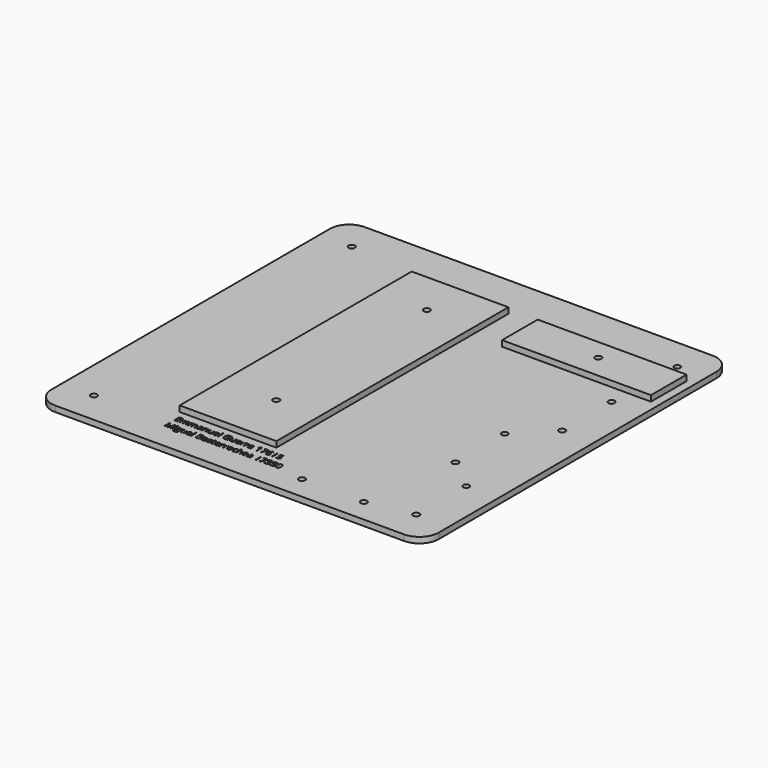
from build123d import *

# Parameters (mm, degrees)
F1_W     = 77
F1_H     = 23
F1_R     = 1.65
F2_DEPTH = 3
F1_W_2   = 50
F1_H_2   = 150
F0_R     = 1.65
F0_W     = 0.3829869529
F0_H     = 2.5274187162
F0_H_2   = 3.5885656107
F0_R_2   = 1.6
F0_R_3   = 1.5699036084
F3_DEPTH = 3


with BuildPart() as f2:
    # F1 (on face) → F2 (new body)
    with BuildSketch(Plane.XY):
        with Locations((51.0507548302, 182.7138311565)):
            Rectangle(F1_W, F1_H)
        with Locations((52.503246814, 183.4763586521)):
            Circle(F1_R, mode=Mode.SUBTRACT)
    extrude(amount=F2_DEPTH)


with BuildPart() as f2b:
    # F1 (on face) → F2, piece 2 (new body)
    with BuildSketch(Plane.XY):
        with Locations((-28.4492451698, 120.280392617)):
            Rectangle(F1_W_2, F1_H_2)
        with Locations((-25.9235966951, 73.280392617)):
            Circle(F1_R, mode=Mode.SUBTRACT)
        with Locations((-27.6105515659, 172.7917194366)):
            Circle(F1_R, mode=Mode.SUBTRACT)
    extrude(amount=F2_DEPTH)


with BuildPart() as f3:
    # F0 (on Top) → F3 (new body)
    with BuildSketch(Plane.XY):
        with BuildLine():
            Line((83.8132826576, 218.280392617), (-96.1867336176, 218.280392617))
            ThreePointArc((-96.1867336176, 218.280392617), (-103.2578014295, 215.3514604289), (-106.1867336176, 208.280392617))
            Line((-106.1867336176, 208.280392617), (-106.1867336176, 28.280392617))
            ThreePointArc((-106.1867336176, 28.280392617), (-103.2578014295, 21.2093248051), (-96.1867336176, 18.280392617))
            Line((-96.1867336176, 18.280392617), (84.1380343496, 18.280392617))
            ThreePointArc((84.1380343496, 18.280392617), (91.2154780023, 21.2157064001), (94.1380180744, 28.2984343483))
            Line((94.1380180744, 28.2984343483), (93.8132663824, 208.2984343483))
            ThreePointArc((93.8132663824, 208.2984343483), (90.8779688745, 215.3578362696), (83.8132826576, 218.280392617))
        make_face()
        with Locations((-89.5367336176, 34.930392617)):
            Circle(F0_R, mode=Mode.SUBTRACT)
        with BuildLine():
            Line((-48.8614755741, 31.815888981), (-49.177310672, 31.815888981))
            Line((-49.177310672, 31.815888981), (-50.3211060034, 34.8045154921))
            Line((-50.3211060034, 34.8045154921), (-50.3395543152, 34.8045154921))
            add(Edge.make_bspline(
                [(-50.3395543152, 34.8045154921), (-50.3070852865, 34.4495699731), (-50.3070852865, 33.9603207443)],
                knots=[0, 0, 0, 1, 1, 1], degree=2))
            Line((-50.3070852865, 33.9603207443), (-50.3070852865, 31.815888981))
            Line((-50.3070852865, 31.815888981), (-50.6694101302, 31.815888981))
            Line((-50.6694101302, 31.815888981), (-50.6694101302, 35.187502445))
            Line((-50.6694101302, 35.187502445), (-50.0790641527, 35.187502445))
            Line((-50.0790641527, 35.187502445), (-49.0112758659, 32.4062349585))
            Line((-49.0112758659, 32.4062349585), (-48.9928275541, 32.4062349585))
            Line((-48.9928275541, 32.4062349585), (-47.9161840776, 35.187502445))
            Line((-47.9161840776, 35.187502445), (-47.330265695, 35.187502445))
            Line((-47.330265695, 35.187502445), (-47.330265695, 31.815888981))
            Line((-47.330265695, 31.815888981), (-47.7221078375, 31.815888981))
            Line((-47.7221078375, 31.815888981), (-47.7221078375, 33.9883621782))
            add(Edge.make_bspline(
                [(-47.7221078375, 33.9883621782), (-47.7221078375, 34.361756009), (-47.6896388088, 34.8000878973)],
                knots=[0, 0, 0, 1, 1, 1], degree=2))
            Line((-47.6896388088, 34.8000878973), (-47.7080871206, 34.8000878973))
            Line((-47.7080871206, 34.8000878973), (-48.8614755741, 31.815888981))
        make_face(mode=Mode.SUBTRACT)
        with Locations((-46.2717015641, 33.0795983391)):
            Rectangle(F0_W, F0_H, mode=Mode.SUBTRACT)
        with BuildLine():
            Line((-44.0737696966, 34.3433076972), (-43.2000576499, 34.3433076972))
            Line((-43.2000576499, 34.3433076972), (-43.2000576499, 34.1012658464))
            Line((-43.2000576499, 34.1012658464), (-43.6679068371, 34.045920911))
            add(Edge.make_bspline(
                [(-43.6679068371, 34.045920911), (-43.603706712, 33.9654862716), (-43.5527893715, 33.8348722241)],
                knots=[0, 0, 0, 1, 1, 1], degree=2))
            add(Edge.make_bspline(
                [(-43.5527893715, 33.8348722241), (-43.5018720309, 33.7042581765), (-43.5018720309, 33.5411751003)],
                knots=[0, 0, 0, 1, 1, 1], degree=2))
            add(Edge.make_bspline(
                [(-43.5018720309, 33.5411751003), (-43.5018720309, 33.1692571344), (-43.7557208012, 32.9478773929)],
                knots=[0, 0, 0, 1, 1, 1], degree=2))
            add(Edge.make_bspline(
                [(-43.7557208012, 32.9478773929), (-44.0095695715, 32.7264976513), (-44.4523290547, 32.7264976513)],
                knots=[0, 0, 0, 1, 1, 1], degree=2))
            add(Edge.make_bspline(
                [(-44.4523290547, 32.7264976513), (-44.5652327229, 32.7264976513), (-44.6641156741, 32.7449459631)],
                knots=[0, 0, 0, 1, 1, 1], degree=2))
            add(Edge.make_bspline(
                [(-44.6641156741, 32.7449459631), (-44.9083713223, 32.6158077805), (-44.9083713223, 32.4202556755)],
                knots=[0, 0, 0, 1, 1, 1], degree=2))
            add(Edge.make_bspline(
                [(-44.9083713223, 32.4202556755), (-44.9083713223, 32.316207197), (-44.8231401218, 32.2667657213)],
                knots=[0, 0, 0, 1, 1, 1], degree=2))
            add(Edge.make_bspline(
                [(-44.8231401218, 32.2667657213), (-44.7379089213, 32.2173242457), (-44.5305498967, 32.2173242457)],
                knots=[0, 0, 0, 1, 1, 1], degree=2))
            Line((-44.5305498967, 32.2173242457), (-44.0833628187, 32.2173242457))
            add(Edge.make_bspline(
                [(-44.0833628187, 32.2173242457), (-43.6723344319, 32.2173242457), (-43.4524305553, 32.0442790811)],
                knots=[0, 0, 0, 1, 1, 1], degree=2))
            add(Edge.make_bspline(
                [(-43.4524305553, 32.0442790811), (-43.2325266787, 31.8712339164), (-43.2325266787, 31.5413781015)],
                knots=[0, 0, 0, 1, 1, 1], degree=2))
            add(Edge.make_bspline(
                [(-43.2325266787, 31.5413781015), (-43.2325266787, 31.121494525), (-43.5690238858, 30.9012216821)],
                knots=[0, 0, 0, 1, 1, 1], degree=2))
            add(Edge.make_bspline(
                [(-43.5690238858, 30.9012216821), (-43.905521093, 30.6809488393), (-44.5512120059, 30.6809488393)],
                knots=[0, 0, 0, 1, 1, 1], degree=2))
            add(Edge.make_bspline(
                [(-44.5512120059, 30.6809488393), (-45.047102627, 30.6809488393), (-45.3157100468, 30.8654319573)],
                knots=[0, 0, 0, 1, 1, 1], degree=2))
            add(Edge.make_bspline(
                [(-45.3157100468, 30.8654319573), (-45.5843174665, 31.0499150752), (-45.5843174665, 31.3871502149)],
                knots=[0, 0, 0, 1, 1, 1], degree=2))
            add(Edge.make_bspline(
                [(-45.5843174665, 31.3871502149), (-45.5843174665, 31.6173851461), (-45.4367309721, 31.7860027159)],
                knots=[0, 0, 0, 1, 1, 1], degree=2))
            add(Edge.make_bspline(
                [(-45.4367309721, 31.7860027159), (-45.2891444778, 31.9546202857), (-45.022012923, 32.014392816)],
                knots=[0, 0, 0, 1, 1, 1], degree=2))
            add(Edge.make_bspline(
                [(-45.022012923, 32.014392816), (-45.1186820768, 32.0579308318), (-45.1843580668, 32.1501723908)],
                knots=[0, 0, 0, 1, 1, 1], degree=2))
            add(Edge.make_bspline(
                [(-45.1843580668, 32.1501723908), (-45.2500340568, 32.2424139498), (-45.2500340568, 32.3649107401)],
                knots=[0, 0, 0, 1, 1, 1], degree=2))
            add(Edge.make_bspline(
                [(-45.2500340568, 32.3649107401), (-45.2500340568, 32.5029041123), (-45.1762408096, 32.6069525909)],
                knots=[0, 0, 0, 1, 1, 1], degree=2))
            add(Edge.make_bspline(
                [(-45.1762408096, 32.6069525909), (-45.1024475624, 32.7110010694), (-44.9430541485, 32.8076702232)],
                knots=[0, 0, 0, 1, 1, 1], degree=2))
            add(Edge.make_bspline(
                [(-44.9430541485, 32.8076702232), (-45.139344186, 32.8881048626), (-45.2625789088, 33.0818121365)],
                knots=[0, 0, 0, 1, 1, 1], degree=2))
            add(Edge.make_bspline(
                [(-45.2625789088, 33.0818121365), (-45.3858136316, 33.2755194104), (-45.3858136316, 33.5249405859)],
                knots=[0, 0, 0, 1, 1, 1], degree=2))
            add(Edge.make_bspline(
                [(-45.3858136316, 33.5249405859), (-45.3858136316, 33.9396586351), (-45.1367614223, 34.164728039)],
                knots=[0, 0, 0, 1, 1, 1], degree=2))
            add(Edge.make_bspline(
                [(-45.1367614223, 34.164728039), (-44.8877092131, 34.3897974429), (-44.4316669455, 34.3897974429)],
                knots=[0, 0, 0, 1, 1, 1], degree=2))
            add(Edge.make_bspline(
                [(-44.4316669455, 34.3897974429), (-44.2331631105, 34.3897974429), (-44.0737696966, 34.3433076972)],
                knots=[0, 0, 0, 1, 1, 1], degree=2))
        make_face(mode=Mode.SUBTRACT)
        with BuildLine():
            add(Edge.make_bspline(
                [(-46.431094978, 34.8355086559), (-46.4956640693, 34.8989708485), (-46.4956640693, 35.0281090311)],
                knots=[0, 0, 0, 1, 1, 1], degree=2))
            add(Edge.make_bspline(
                [(-46.4956640693, 35.0281090311), (-46.4956640693, 35.1594610111), (-46.431094978, 35.2207094062)],
                knots=[0, 0, 0, 1, 1, 1], degree=2))
            add(Edge.make_bspline(
                [(-46.431094978, 35.2207094062), (-46.3665258867, 35.2819578014), (-46.2691188004, 35.2819578014)],
                knots=[0, 0, 0, 1, 1, 1], degree=2))
            add(Edge.make_bspline(
                [(-46.2691188004, 35.2819578014), (-46.1768772414, 35.2819578014), (-46.1100943527, 35.2196025075)],
                knots=[0, 0, 0, 1, 1, 1], degree=2))
            add(Edge.make_bspline(
                [(-46.1100943527, 35.2196025075), (-46.043311464, 35.1572472136), (-46.043311464, 35.0281090311)],
                knots=[0, 0, 0, 1, 1, 1], degree=2))
            add(Edge.make_bspline(
                [(-46.043311464, 35.0281090311), (-46.043311464, 34.8989708485), (-46.1100943527, 34.8355086559)],
                knots=[0, 0, 0, 1, 1, 1], degree=2))
            add(Edge.make_bspline(
                [(-46.1100943527, 34.8355086559), (-46.1768772414, 34.7720464633), (-46.2691188004, 34.7720464633)],
                knots=[0, 0, 0, 1, 1, 1], degree=2))
            add(Edge.make_bspline(
                [(-46.2691188004, 34.7720464633), (-46.3665258867, 34.7720464633), (-46.431094978, 34.8355086559)],
                knots=[0, 0, 0, 1, 1, 1], degree=2))
        make_face(mode=Mode.SUBTRACT)
        Polygon((-48.7898961243, 38.5893711403), (-48.7898961243, 38.2388532162), (-50.6694101302, 38.2388532162), (-50.6694101302, 41.6104666801), (-48.7898961243, 41.6104666801), (-48.7898961243, 41.2621625534), (-50.2775679876, 41.2621625534), (-50.2775679876, 40.1759259548), (-48.8799238859, 40.1759259548), (-48.8799238859, 39.8298356255), (-50.2775679876, 39.8298356255), (-50.2775679876, 38.5893711403), align=None, mode=Mode.SUBTRACT)
        with BuildLine():
            Line((-44.496605003, 38.2388532162), (-44.8788540234, 38.2388532162))
            Line((-44.8788540234, 38.2388532162), (-44.8788540234, 39.8829667635))
            add(Edge.make_bspline(
                [(-44.8788540234, 39.8829667635), (-44.8788540234, 40.185519077), (-45.007992206, 40.3364262675)],
                knots=[0, 0, 0, 1, 1, 1], degree=2))
            add(Edge.make_bspline(
                [(-45.007992206, 40.3364262675), (-45.1371303886, 40.487333458), (-45.4094274707, 40.487333458)],
                knots=[0, 0, 0, 1, 1, 1], degree=2))
            add(Edge.make_bspline(
                [(-45.4094274707, 40.487333458), (-45.7665867871, 40.487333458), (-45.9374181543, 40.2821882308)],
                knots=[0, 0, 0, 1, 1, 1], degree=2))
            add(Edge.make_bspline(
                [(-45.9374181543, 40.2821882308), (-46.1082495215, 40.0770430036), (-46.1082495215, 39.6505180349)],
                knots=[0, 0, 0, 1, 1, 1], degree=2))
            Line((-46.1082495215, 39.6505180349), (-46.1082495215, 38.2388532162))
            Line((-46.1082495215, 38.2388532162), (-46.4912364744, 38.2388532162))
            Line((-46.4912364744, 38.2388532162), (-46.4912364744, 39.8829667635))
            add(Edge.make_bspline(
                [(-46.4912364744, 39.8829667635), (-46.4912364744, 40.185519077), (-46.620374657, 40.3364262675)],
                knots=[0, 0, 0, 1, 1, 1], degree=2))
            add(Edge.make_bspline(
                [(-46.620374657, 40.3364262675), (-46.7495128396, 40.487333458), (-47.0240237191, 40.487333458)],
                knots=[0, 0, 0, 1, 1, 1], degree=2))
            add(Edge.make_bspline(
                [(-47.0240237191, 40.487333458), (-47.3833968329, 40.487333458), (-47.5505385378, 40.2718571762)],
                knots=[0, 0, 0, 1, 1, 1], degree=2))
            add(Edge.make_bspline(
                [(-47.5505385378, 40.2718571762), (-47.7176802427, 40.0563808944), (-47.7176802427, 39.5649178681)],
                knots=[0, 0, 0, 1, 1, 1], degree=2))
            Line((-47.7176802427, 39.5649178681), (-47.7176802427, 38.2388532162))
            Line((-47.7176802427, 38.2388532162), (-48.1006671956, 38.2388532162))
            Line((-48.1006671956, 38.2388532162), (-48.1006671956, 40.7662719323))
            Line((-48.1006671956, 40.7662719323), (-47.7892596925, 40.7662719323))
            Line((-47.7892596925, 40.7662719323), (-47.7272733648, 40.420181603))
            Line((-47.7272733648, 40.420181603), (-47.708825053, 40.420181603))
            add(Edge.make_bspline(
                [(-47.708825053, 40.420181603), (-47.6003489797, 40.604664721), (-47.4029520434, 40.7087131995)],
                knots=[0, 0, 0, 1, 1, 1], degree=2))
            add(Edge.make_bspline(
                [(-47.4029520434, 40.7087131995), (-47.2055551072, 40.812761678), (-46.961299459, 40.812761678)],
                knots=[0, 0, 0, 1, 1, 1], degree=2))
            add(Edge.make_bspline(
                [(-46.961299459, 40.812761678), (-46.3687396841, 40.812761678), (-46.1864703636, 40.3832849794)],
                knots=[0, 0, 0, 1, 1, 1], degree=2))
            Line((-46.1864703636, 40.3832849794), (-46.1680220518, 40.3832849794))
            add(Edge.make_bspline(
                [(-46.1680220518, 40.3832849794), (-46.0551183836, 40.5817888144), (-45.8407490005, 40.6972752462)],
                knots=[0, 0, 0, 1, 1, 1], degree=2))
            add(Edge.make_bspline(
                [(-45.8407490005, 40.6972752462), (-45.6263796174, 40.812761678), (-45.3518687379, 40.812761678)],
                knots=[0, 0, 0, 1, 1, 1], degree=2))
            add(Edge.make_bspline(
                [(-45.3518687379, 40.812761678), (-44.9231299717, 40.812761678), (-44.7098674874, 40.5924888352)],
                knots=[0, 0, 0, 1, 1, 1], degree=2))
            add(Edge.make_bspline(
                [(-44.7098674874, 40.5924888352), (-44.496605003, 40.3722159923), (-44.496605003, 39.8873943583)],
                knots=[0, 0, 0, 1, 1, 1], degree=2))
            Line((-44.496605003, 39.8873943583), (-44.496605003, 38.2388532162))
        make_face(mode=Mode.SUBTRACT)
        with BuildLine():
            Line((-42.7085946236, 34.3433076972), (-42.3211800759, 34.3433076972))
            Line((-42.3211800759, 34.3433076972), (-42.3211800759, 32.7036217447))
            add(Edge.make_bspline(
                [(-42.3211800759, 32.7036217447), (-42.3211800759, 32.394428039), (-42.18060394, 32.2424139498)],
                knots=[0, 0, 0, 1, 1, 1], degree=2))
            add(Edge.make_bspline(
                [(-42.18060394, 32.2424139498), (-42.0400278041, 32.0903998606), (-41.7404272206, 32.0903998606)],
                knots=[0, 0, 0, 1, 1, 1], degree=2))
            add(Edge.make_bspline(
                [(-41.7404272206, 32.0903998606), (-41.3434195507, 32.0903998606), (-41.1604122977, 32.3069830411)],
                knots=[0, 0, 0, 1, 1, 1], degree=2))
            add(Edge.make_bspline(
                [(-41.1604122977, 32.3069830411), (-40.9774050446, 32.5235662215), (-40.9774050446, 33.0150292478)],
                knots=[0, 0, 0, 1, 1, 1], degree=2))
            Line((-40.9774050446, 33.0150292478), (-40.9774050446, 34.3433076972))
            Line((-40.9774050446, 34.3433076972), (-40.5944180917, 34.3433076972))
            Line((-40.5944180917, 34.3433076972), (-40.5944180917, 31.815888981))
            Line((-40.5944180917, 31.815888981), (-40.9102531897, 31.815888981))
            Line((-40.9102531897, 31.815888981), (-40.9655981251, 32.1545999856))
            Line((-40.9655981251, 32.1545999856), (-40.9862602343, 32.1545999856))
            add(Edge.make_bspline(
                [(-40.9862602343, 32.1545999856), (-41.1035914973, 31.9679030702), (-41.3124263869, 31.8686511528)],
                knots=[0, 0, 0, 1, 1, 1], degree=2))
            add(Edge.make_bspline(
                [(-41.3124263869, 31.8686511528), (-41.5212612764, 31.7693992353), (-41.7891307637, 31.7693992353)],
                knots=[0, 0, 0, 1, 1, 1], degree=2))
            add(Edge.make_bspline(
                [(-41.7891307637, 31.7693992353), (-42.2503385586, 31.7693992353), (-42.4794665911, 31.9885651794)],
                knots=[0, 0, 0, 1, 1, 1], degree=2))
            add(Edge.make_bspline(
                [(-42.4794665911, 31.9885651794), (-42.7085946236, 32.2077311236), (-42.7085946236, 32.6896010277)],
                knots=[0, 0, 0, 1, 1, 1], degree=2))
            Line((-42.7085946236, 32.6896010277), (-42.7085946236, 34.3433076972))
        make_face(mode=Mode.SUBTRACT)
        with BuildLine():
            add(Edge.make_bspline(
                [(-38.2780480625, 31.8077717238), (-38.4588415181, 31.7693992353), (-38.7149040859, 31.7693992353)],
                knots=[0, 0, 0, 1, 1, 1], degree=2))
            add(Edge.make_bspline(
                [(-38.7149040859, 31.7693992353), (-39.274994832, 31.7693992353), (-39.5993161534, 32.1110619698)],
                knots=[0, 0, 0, 1, 1, 1], degree=2))
            add(Edge.make_bspline(
                [(-39.5993161534, 32.1110619698), (-39.9236374748, 32.4527247042), (-39.9236374748, 33.0585672637)],
                knots=[0, 0, 0, 1, 1, 1], degree=2))
            add(Edge.make_bspline(
                [(-39.9236374748, 33.0585672637), (-39.9236374748, 33.6703132828), (-39.6225610263, 34.0300553629)],
                knots=[0, 0, 0, 1, 1, 1], degree=2))
            add(Edge.make_bspline(
                [(-39.6225610263, 34.0300553629), (-39.3214845778, 34.3897974429), (-38.8137870371, 34.3897974429)],
                knots=[0, 0, 0, 1, 1, 1], degree=2))
            add(Edge.make_bspline(
                [(-38.8137870371, 34.3897974429), (-38.3392964577, 34.3897974429), (-38.0625717808, 34.0772830411)],
                knots=[0, 0, 0, 1, 1, 1], degree=2))
            add(Edge.make_bspline(
                [(-38.0625717808, 34.0772830411), (-37.7858471038, 33.7647686392), (-37.7858471038, 33.2526435038)],
                knots=[0, 0, 0, 1, 1, 1], degree=2))
            Line((-37.7858471038, 33.2526435038), (-37.7858471038, 33.010601653))
            Line((-37.7858471038, 33.010601653), (-39.5266298049, 33.010601653))
            add(Edge.make_bspline(
                [(-39.5266298049, 33.010601653), (-39.5148228854, 32.5656283724), (-39.301560401, 32.335024475)],
                knots=[0, 0, 0, 1, 1, 1], degree=2))
            add(Edge.make_bspline(
                [(-39.301560401, 32.335024475), (-39.0882979167, 32.1044205775), (-38.7008833689, 32.1044205775)],
                knots=[0, 0, 0, 1, 1, 1], degree=2))
            add(Edge.make_bspline(
                [(-38.7008833689, 32.1044205775), (-38.292806712, 32.1044205775), (-37.8943231772, 32.2748829785)],
                knots=[0, 0, 0, 1, 1, 1], degree=2))
            Line((-37.8943231772, 32.2748829785), (-37.8943231772, 31.9332202441))
            add(Edge.make_bspline(
                [(-37.8943231772, 31.9332202441), (-38.0972546069, 31.8461442124), (-38.2780480625, 31.8077717238)],
                knots=[0, 0, 0, 1, 1, 1], degree=2))
        make_face(mode=Mode.SUBTRACT)
        with Locations((-36.9412833898, 33.6101717864)):
            Rectangle(F0_W, F0_H_2, mode=Mode.SUBTRACT)
        with BuildLine():
            Line((-34.6533237607, 31.815888981), (-34.6533237607, 35.187502445))
            Line((-34.6533237607, 35.187502445), (-33.7006529395, 35.187502445))
            add(Edge.make_bspline(
                [(-33.7006529395, 35.187502445), (-33.0298723226, 35.187502445), (-32.7299027728, 34.9867848126)],
                knots=[0, 0, 0, 1, 1, 1], degree=2))
            add(Edge.make_bspline(
                [(-32.7299027728, 34.9867848126), (-32.429933223, 34.7860671803), (-32.429933223, 34.3529008193)],
                knots=[0, 0, 0, 1, 1, 1], degree=2))
            add(Edge.make_bspline(
                [(-32.429933223, 34.3529008193), (-32.429933223, 34.0525623033), (-32.5970749279, 33.8577481307)],
                knots=[0, 0, 0, 1, 1, 1], degree=2))
            add(Edge.make_bspline(
                [(-32.5970749279, 33.8577481307), (-32.7642166327, 33.6629339581), (-33.085217258, 33.6053752253)],
                knots=[0, 0, 0, 1, 1, 1], degree=2))
            Line((-33.085217258, 33.6053752253), (-33.085217258, 33.5824993187))
            add(Edge.make_bspline(
                [(-33.085217258, 33.5824993187), (-32.3170295548, 33.4511473387), (-32.3170295548, 32.7752011945)],
                knots=[0, 0, 0, 1, 1, 1], degree=2))
            add(Edge.make_bspline(
                [(-32.3170295548, 32.7752011945), (-32.3170295548, 32.3235865217), (-32.6225335981, 32.0697377513)],
                knots=[0, 0, 0, 1, 1, 1], degree=2))
            add(Edge.make_bspline(
                [(-32.6225335981, 32.0697377513), (-32.9280376415, 31.815888981), (-33.4770594006, 31.815888981)],
                knots=[0, 0, 0, 1, 1, 1], degree=2))
            Line((-33.4770594006, 31.815888981), (-34.6533237607, 31.815888981))
        make_face(mode=Mode.SUBTRACT)
        with BuildLine():
            Line((-40.1036929979, 38.2388532162), (-40.4859420184, 38.2388532162))
            Line((-40.4859420184, 38.2388532162), (-40.4859420184, 39.8829667635))
            add(Edge.make_bspline(
                [(-40.4859420184, 39.8829667635), (-40.4859420184, 40.185519077), (-40.615080201, 40.3364262675)],
                knots=[0, 0, 0, 1, 1, 1], degree=2))
            add(Edge.make_bspline(
                [(-40.615080201, 40.3364262675), (-40.7442183835, 40.487333458), (-41.0165154656, 40.487333458)],
                knots=[0, 0, 0, 1, 1, 1], degree=2))
            add(Edge.make_bspline(
                [(-41.0165154656, 40.487333458), (-41.373674782, 40.487333458), (-41.5445061493, 40.2821882308)],
                knots=[0, 0, 0, 1, 1, 1], degree=2))
            add(Edge.make_bspline(
                [(-41.5445061493, 40.2821882308), (-41.7153375165, 40.0770430036), (-41.7153375165, 39.6505180349)],
                knots=[0, 0, 0, 1, 1, 1], degree=2))
            Line((-41.7153375165, 39.6505180349), (-41.7153375165, 38.2388532162))
            Line((-41.7153375165, 38.2388532162), (-42.0983244694, 38.2388532162))
            Line((-42.0983244694, 38.2388532162), (-42.0983244694, 39.8829667635))
            add(Edge.make_bspline(
                [(-42.0983244694, 39.8829667635), (-42.0983244694, 40.185519077), (-42.227462652, 40.3364262675)],
                knots=[0, 0, 0, 1, 1, 1], degree=2))
            add(Edge.make_bspline(
                [(-42.227462652, 40.3364262675), (-42.3566008346, 40.487333458), (-42.6311117141, 40.487333458)],
                knots=[0, 0, 0, 1, 1, 1], degree=2))
            add(Edge.make_bspline(
                [(-42.6311117141, 40.487333458), (-42.9904848279, 40.487333458), (-43.1576265328, 40.2718571762)],
                knots=[0, 0, 0, 1, 1, 1], degree=2))
            add(Edge.make_bspline(
                [(-43.1576265328, 40.2718571762), (-43.3247682377, 40.0563808944), (-43.3247682377, 39.5649178681)],
                knots=[0, 0, 0, 1, 1, 1], degree=2))
            Line((-43.3247682377, 39.5649178681), (-43.3247682377, 38.2388532162))
            Line((-43.3247682377, 38.2388532162), (-43.7077551906, 38.2388532162))
            Line((-43.7077551906, 38.2388532162), (-43.7077551906, 40.7662719323))
            Line((-43.7077551906, 40.7662719323), (-43.3963476874, 40.7662719323))
            Line((-43.3963476874, 40.7662719323), (-43.3343613598, 40.420181603))
            Line((-43.3343613598, 40.420181603), (-43.315913048, 40.420181603))
            add(Edge.make_bspline(
                [(-43.315913048, 40.420181603), (-43.2074369746, 40.604664721), (-43.0100400384, 40.7087131995)],
                knots=[0, 0, 0, 1, 1, 1], degree=2))
            add(Edge.make_bspline(
                [(-43.0100400384, 40.7087131995), (-42.8126431022, 40.812761678), (-42.568387454, 40.812761678)],
                knots=[0, 0, 0, 1, 1, 1], degree=2))
            add(Edge.make_bspline(
                [(-42.568387454, 40.812761678), (-41.9758276791, 40.812761678), (-41.7935583585, 40.3832849794)],
                knots=[0, 0, 0, 1, 1, 1], degree=2))
            Line((-41.7935583585, 40.3832849794), (-41.7751100467, 40.3832849794))
            add(Edge.make_bspline(
                [(-41.7751100467, 40.3832849794), (-41.6622063785, 40.5817888144), (-41.4478369955, 40.6972752462)],
                knots=[0, 0, 0, 1, 1, 1], degree=2))
            add(Edge.make_bspline(
                [(-41.4478369955, 40.6972752462), (-41.2334676124, 40.812761678), (-40.9589567328, 40.812761678)],
                knots=[0, 0, 0, 1, 1, 1], degree=2))
            add(Edge.make_bspline(
                [(-40.9589567328, 40.812761678), (-40.5302179667, 40.812761678), (-40.3169554823, 40.5924888352)],
                knots=[0, 0, 0, 1, 1, 1], degree=2))
            add(Edge.make_bspline(
                [(-40.3169554823, 40.5924888352), (-40.1036929979, 40.3722159923), (-40.1036929979, 39.8873943583)],
                knots=[0, 0, 0, 1, 1, 1], degree=2))
            Line((-40.1036929979, 39.8873943583), (-40.1036929979, 38.2388532162))
        make_face(mode=Mode.SUBTRACT)
        with BuildLine():
            Line((-37.4766533981, 38.2388532162), (-37.7607573998, 38.2388532162))
            Line((-37.7607573998, 38.2388532162), (-37.8367644444, 38.5989642624))
            Line((-37.8367644444, 38.5989642624), (-37.8552127562, 38.5989642624))
            add(Edge.make_bspline(
                [(-37.8552127562, 38.5989642624), (-38.044123469, 38.3613500065), (-38.2319272831, 38.2768567385)],
                knots=[0, 0, 0, 1, 1, 1], degree=2))
            add(Edge.make_bspline(
                [(-38.2319272831, 38.2768567385), (-38.4197310971, 38.1923634704), (-38.7016213014, 38.1923634704)],
                knots=[0, 0, 0, 1, 1, 1], degree=2))
            add(Edge.make_bspline(
                [(-38.7016213014, 38.1923634704), (-39.0772289296, 38.1923634704), (-39.2904914139, 38.3864397105)],
                knots=[0, 0, 0, 1, 1, 1], degree=2))
            add(Edge.make_bspline(
                [(-39.2904914139, 38.3864397105), (-39.5037538983, 38.5805159506), (-39.5037538983, 38.937675267)],
                knots=[0, 0, 0, 1, 1, 1], degree=2))
            add(Edge.make_bspline(
                [(-39.5037538983, 38.937675267), (-39.5037538983, 39.7029112404), (-38.2795239275, 39.739807864)],
                knots=[0, 0, 0, 1, 1, 1], degree=2))
            Line((-38.2795239275, 39.739807864), (-37.8507851613, 39.7538285809))
            Line((-37.8507851613, 39.7538285809), (-37.8507851613, 39.9110081974))
            add(Edge.make_bspline(
                [(-37.8507851613, 39.9110081974), (-37.8507851613, 40.2083949836), (-37.978447479, 40.3500780182)],
                knots=[0, 0, 0, 1, 1, 1], degree=2))
            add(Edge.make_bspline(
                [(-37.978447479, 40.3500780182), (-38.1061097966, 40.4917610528), (-38.3880000009, 40.4917610528)],
                knots=[0, 0, 0, 1, 1, 1], degree=2))
            add(Edge.make_bspline(
                [(-38.3880000009, 40.4917610528), (-38.7038350988, 40.4917610528), (-39.1023186336, 40.2984227452)],
                knots=[0, 0, 0, 1, 1, 1], degree=2))
            Line((-39.1023186336, 40.2984227452), (-39.2203878291, 40.5913819365))
            add(Edge.make_bspline(
                [(-39.2203878291, 40.5913819365), (-39.0336909137, 40.6924786851), (-38.8112042735, 40.7500374179)],
                knots=[0, 0, 0, 1, 1, 1], degree=2))
            add(Edge.make_bspline(
                [(-38.8112042735, 40.7500374179), (-38.5887176332, 40.8075961507), (-38.3643861618, 40.8075961507)],
                knots=[0, 0, 0, 1, 1, 1], degree=2))
            add(Edge.make_bspline(
                [(-38.3643861618, 40.8075961507), (-37.912771489, 40.8075961507), (-37.6947124435, 40.6072474846)],
                knots=[0, 0, 0, 1, 1, 1], degree=2))
            add(Edge.make_bspline(
                [(-37.6947124435, 40.6072474846), (-37.4766533981, 40.4068988185), (-37.4766533981, 39.9641393354)],
                knots=[0, 0, 0, 1, 1, 1], degree=2))
            Line((-37.4766533981, 39.9641393354), (-37.4766533981, 38.2388532162))
        make_face(mode=Mode.SUBTRACT)
        with BuildLine():
            Line((-34.5758408512, 38.2388532162), (-34.9588278041, 38.2388532162))
            Line((-34.9588278041, 38.2388532162), (-34.9588278041, 39.8741115738))
            add(Edge.make_bspline(
                [(-34.9588278041, 39.8741115738), (-34.9588278041, 40.1825673471), (-35.09940394, 40.3349504025)],
                knots=[0, 0, 0, 1, 1, 1], degree=2))
            add(Edge.make_bspline(
                [(-35.09940394, 40.3349504025), (-35.2399800759, 40.487333458), (-35.5403185919, 40.487333458)],
                knots=[0, 0, 0, 1, 1, 1], degree=2))
            add(Edge.make_bspline(
                [(-35.5403185919, 40.487333458), (-35.9365883293, 40.487333458), (-36.1210714473, 40.2729640749)],
                knots=[0, 0, 0, 1, 1, 1], degree=2))
            add(Edge.make_bspline(
                [(-36.1210714473, 40.2729640749), (-36.3055545652, 40.0585946918), (-36.3055545652, 39.5649178681)],
                knots=[0, 0, 0, 1, 1, 1], degree=2))
            Line((-36.3055545652, 39.5649178681), (-36.3055545652, 38.2388532162))
            Line((-36.3055545652, 38.2388532162), (-36.6885415181, 38.2388532162))
            Line((-36.6885415181, 38.2388532162), (-36.6885415181, 40.7662719323))
            Line((-36.6885415181, 40.7662719323), (-36.377134015, 40.7662719323))
            Line((-36.377134015, 40.7662719323), (-36.3151476874, 40.420181603))
            Line((-36.3151476874, 40.420181603), (-36.2966993756, 40.420181603))
            add(Edge.make_bspline(
                [(-36.2966993756, 40.420181603), (-36.1786301801, 40.6068785184), (-35.9664745944, 40.7098200982)],
                knots=[0, 0, 0, 1, 1, 1], degree=2))
            add(Edge.make_bspline(
                [(-35.9664745944, 40.7098200982), (-35.7543190088, 40.812761678), (-35.4938288462, 40.812761678)],
                knots=[0, 0, 0, 1, 1, 1], degree=2))
            add(Edge.make_bspline(
                [(-35.4938288462, 40.812761678), (-35.0370486461, 40.812761678), (-34.8064447486, 40.5924888352)],
                knots=[0, 0, 0, 1, 1, 1], degree=2))
            add(Edge.make_bspline(
                [(-34.8064447486, 40.5924888352), (-34.5758408512, 40.3722159923), (-34.5758408512, 39.8873943583)],
                knots=[0, 0, 0, 1, 1, 1], degree=2))
            Line((-34.5758408512, 39.8873943583), (-34.5758408512, 38.2388532162))
        make_face(mode=Mode.SUBTRACT)
        with BuildLine():
            Line((-33.8172462701, 40.7662719323), (-33.4298317224, 40.7662719323))
            Line((-33.4298317224, 40.7662719323), (-33.4298317224, 39.1265859798))
            add(Edge.make_bspline(
                [(-33.4298317224, 39.1265859798), (-33.4298317224, 38.8173922741), (-33.2892555865, 38.6653781849)],
                knots=[0, 0, 0, 1, 1, 1], degree=2))
            add(Edge.make_bspline(
                [(-33.2892555865, 38.6653781849), (-33.1486794506, 38.5133640957), (-32.849078867, 38.5133640957)],
                knots=[0, 0, 0, 1, 1, 1], degree=2))
            add(Edge.make_bspline(
                [(-32.849078867, 38.5133640957), (-32.4520711971, 38.5133640957), (-32.2690639441, 38.7299472762)],
                knots=[0, 0, 0, 1, 1, 1], degree=2))
            add(Edge.make_bspline(
                [(-32.2690639441, 38.7299472762), (-32.0860566911, 38.9465304567), (-32.0860566911, 39.437993483)],
                knots=[0, 0, 0, 1, 1, 1], degree=2))
            Line((-32.0860566911, 39.437993483), (-32.0860566911, 40.7662719323))
            Line((-32.0860566911, 40.7662719323), (-31.7030697382, 40.7662719323))
            Line((-31.7030697382, 40.7662719323), (-31.7030697382, 38.2388532162))
            Line((-31.7030697382, 38.2388532162), (-32.0189048361, 38.2388532162))
            Line((-32.0189048361, 38.2388532162), (-32.0742497715, 38.5775642208))
            Line((-32.0742497715, 38.5775642208), (-32.0949118808, 38.5775642208))
            add(Edge.make_bspline(
                [(-32.0949118808, 38.5775642208), (-32.2122431438, 38.3908673054), (-32.4210780333, 38.2916153879)],
                knots=[0, 0, 0, 1, 1, 1], degree=2))
            add(Edge.make_bspline(
                [(-32.4210780333, 38.2916153879), (-32.6299129229, 38.1923634704), (-32.8977824101, 38.1923634704)],
                knots=[0, 0, 0, 1, 1, 1], degree=2))
            add(Edge.make_bspline(
                [(-32.8977824101, 38.1923634704), (-33.3589902051, 38.1923634704), (-33.5881182376, 38.4115294146)],
                knots=[0, 0, 0, 1, 1, 1], degree=2))
            add(Edge.make_bspline(
                [(-33.5881182376, 38.4115294146), (-33.8172462701, 38.6306953587), (-33.8172462701, 39.1125652629)],
                knots=[0, 0, 0, 1, 1, 1], degree=2))
            Line((-33.8172462701, 39.1125652629), (-33.8172462701, 40.7662719323))
        make_face(mode=Mode.SUBTRACT)
        with BuildLine():
            Line((-29.8124867453, 31.815888981), (-30.0965907469, 31.815888981))
            Line((-30.0965907469, 31.815888981), (-30.1725977915, 32.1760000273))
            Line((-30.1725977915, 32.1760000273), (-30.1910461033, 32.1760000273))
            add(Edge.make_bspline(
                [(-30.1910461033, 32.1760000273), (-30.3799568161, 31.9383857714), (-30.5677606302, 31.8538925033)],
                knots=[0, 0, 0, 1, 1, 1], degree=2))
            add(Edge.make_bspline(
                [(-30.5677606302, 31.8538925033), (-30.7555644443, 31.7693992353), (-31.0374546486, 31.7693992353)],
                knots=[0, 0, 0, 1, 1, 1], degree=2))
            add(Edge.make_bspline(
                [(-31.0374546486, 31.7693992353), (-31.4130622767, 31.7693992353), (-31.6263247611, 31.9634754754)],
                knots=[0, 0, 0, 1, 1, 1], degree=2))
            add(Edge.make_bspline(
                [(-31.6263247611, 31.9634754754), (-31.8395872455, 32.1575517155), (-31.8395872455, 32.5147110319)],
                knots=[0, 0, 0, 1, 1, 1], degree=2))
            add(Edge.make_bspline(
                [(-31.8395872455, 32.5147110319), (-31.8395872455, 33.2799470052), (-30.6153572747, 33.3168436288)],
                knots=[0, 0, 0, 1, 1, 1], degree=2))
            Line((-30.6153572747, 33.3168436288), (-30.1866185085, 33.3308643458))
            Line((-30.1866185085, 33.3308643458), (-30.1866185085, 33.4880439623))
            add(Edge.make_bspline(
                [(-30.1866185085, 33.4880439623), (-30.1866185085, 33.7854307484), (-30.3142808261, 33.927113783)],
                knots=[0, 0, 0, 1, 1, 1], degree=2))
            add(Edge.make_bspline(
                [(-30.3142808261, 33.927113783), (-30.4419431438, 34.0687968176), (-30.723833348, 34.0687968176)],
                knots=[0, 0, 0, 1, 1, 1], degree=2))
            add(Edge.make_bspline(
                [(-30.723833348, 34.0687968176), (-31.039668446, 34.0687968176), (-31.4381519808, 33.87545851)],
                knots=[0, 0, 0, 1, 1, 1], degree=2))
            Line((-31.4381519808, 33.87545851), (-31.5562211763, 34.1684177013))
            add(Edge.make_bspline(
                [(-31.5562211763, 34.1684177013), (-31.3695242609, 34.26951445), (-31.1470376206, 34.3270731828)],
                knots=[0, 0, 0, 1, 1, 1], degree=2))
            add(Edge.make_bspline(
                [(-31.1470376206, 34.3270731828), (-30.9245509804, 34.3846319156), (-30.7002195089, 34.3846319156)],
                knots=[0, 0, 0, 1, 1, 1], degree=2))
            add(Edge.make_bspline(
                [(-30.7002195089, 34.3846319156), (-30.2486048361, 34.3846319156), (-30.0305457907, 34.1842832495)],
                knots=[0, 0, 0, 1, 1, 1], degree=2))
            add(Edge.make_bspline(
                [(-30.0305457907, 34.1842832495), (-29.8124867453, 33.9839345834), (-29.8124867453, 33.5411751003)],
                knots=[0, 0, 0, 1, 1, 1], degree=2))
            Line((-29.8124867453, 33.5411751003), (-29.8124867453, 31.815888981))
        make_face(mode=Mode.SUBTRACT)
        with BuildLine():
            add(Edge.make_bspline(
                [(-27.5521995839, 32.9227876888), (-27.3942820349, 32.7567528827), (-27.3942820349, 32.5051179097)],
                knots=[0, 0, 0, 1, 1, 1], degree=2))
            add(Edge.make_bspline(
                [(-27.3942820349, 32.5051179097), (-27.3942820349, 32.1523861882), (-27.6569859949, 31.9608927117)],
                knots=[0, 0, 0, 1, 1, 1], degree=2))
            add(Edge.make_bspline(
                [(-27.6569859949, 31.9608927117), (-27.9196899549, 31.7693992353), (-28.3949184668, 31.7693992353)],
                knots=[0, 0, 0, 1, 1, 1], degree=2))
            add(Edge.make_bspline(
                [(-28.3949184668, 31.7693992353), (-28.8974504801, 31.7693992353), (-29.1786027519, 31.9287926492)],
                knots=[0, 0, 0, 1, 1, 1], degree=2))
            Line((-29.1786027519, 31.9287926492), (-29.1786027519, 32.2837381682))
            add(Edge.make_bspline(
                [(-29.1786027519, 32.2837381682), (-28.9963334314, 32.1914966092), (-28.7878675081, 32.1387344375)],
                knots=[0, 0, 0, 1, 1, 1], degree=2))
            add(Edge.make_bspline(
                [(-28.7878675081, 32.1387344375), (-28.5794015848, 32.0859722657), (-28.3853253447, 32.0859722657)],
                knots=[0, 0, 0, 1, 1, 1], degree=2))
            add(Edge.make_bspline(
                [(-28.3853253447, 32.0859722657), (-28.0857247611, 32.0859722657), (-27.924486516, 32.1815345208)],
                knots=[0, 0, 0, 1, 1, 1], degree=2))
            add(Edge.make_bspline(
                [(-27.924486516, 32.1815345208), (-27.7632482709, 32.2770967759), (-27.7632482709, 32.4733868135)],
                knots=[0, 0, 0, 1, 1, 1], degree=2))
            add(Edge.make_bspline(
                [(-27.7632482709, 32.4733868135), (-27.7632482709, 32.6209733078), (-27.8909105885, 32.7257597188)],
                knots=[0, 0, 0, 1, 1, 1], degree=2))
            add(Edge.make_bspline(
                [(-27.8909105885, 32.7257597188), (-28.0185729061, 32.8305461298), (-28.390490872, 32.9737050294)],
                knots=[0, 0, 0, 1, 1, 1], degree=2))
            add(Edge.make_bspline(
                [(-28.390490872, 32.9737050294), (-28.7432225935, 33.1050570094), (-28.8919159866, 33.2032020281)],
                knots=[0, 0, 0, 1, 1, 1], degree=2))
            add(Edge.make_bspline(
                [(-28.8919159866, 33.2032020281), (-29.0406093797, 33.3013470469), (-29.1132957282, 33.4256886684)],
                knots=[0, 0, 0, 1, 1, 1], degree=2))
            add(Edge.make_bspline(
                [(-29.1132957282, 33.4256886684), (-29.1859820766, 33.5500302899), (-29.1859820766, 33.7227064883)],
                knots=[0, 0, 0, 1, 1, 1], degree=2))
            add(Edge.make_bspline(
                [(-29.1859820766, 33.7227064883), (-29.1859820766, 34.031900194), (-28.9343471037, 34.2108488185)],
                knots=[0, 0, 0, 1, 1, 1], degree=2))
            add(Edge.make_bspline(
                [(-28.9343471037, 34.2108488185), (-28.6827121308, 34.3897974429), (-28.245118175, 34.3897974429)],
                knots=[0, 0, 0, 1, 1, 1], degree=2))
            add(Edge.make_bspline(
                [(-28.245118175, 34.3897974429), (-27.8370415181, 34.3897974429), (-27.4466752405, 34.2237626367)],
                knots=[0, 0, 0, 1, 1, 1], degree=2))
            Line((-27.4466752405, 34.2237626367), (-27.5831927477, 33.9123551336))
            add(Edge.make_bspline(
                [(-27.5831927477, 33.9123551336), (-27.9632279708, 34.0687968176), (-28.2724216765, 34.0687968176)],
                knots=[0, 0, 0, 1, 1, 1], degree=2))
            add(Edge.make_bspline(
                [(-28.2724216765, 34.0687968176), (-28.5447187586, 34.0687968176), (-28.6830810971, 33.9835656171)],
                knots=[0, 0, 0, 1, 1, 1], degree=2))
            add(Edge.make_bspline(
                [(-28.6830810971, 33.9835656171), (-28.8214434355, 33.8983344166), (-28.8214434355, 33.7485341248)],
                knots=[0, 0, 0, 1, 1, 1], degree=2))
            add(Edge.make_bspline(
                [(-28.8214434355, 33.7485341248), (-28.8214434355, 33.6466994437), (-28.7694191963, 33.5754889602)],
                knots=[0, 0, 0, 1, 1, 1], degree=2))
            add(Edge.make_bspline(
                [(-28.7694191963, 33.5754889602), (-28.717394957, 33.5042784767), (-28.6022774914, 33.4397093854)],
                knots=[0, 0, 0, 1, 1, 1], degree=2))
            add(Edge.make_bspline(
                [(-28.6022774914, 33.4397093854), (-28.4871600258, 33.3751402941), (-28.1595180083, 33.2526435038)],
                knots=[0, 0, 0, 1, 1, 1], degree=2))
            add(Edge.make_bspline(
                [(-28.1595180083, 33.2526435038), (-27.7101171329, 33.088822495), (-27.5521995839, 32.9227876888)],
                knots=[0, 0, 0, 1, 1, 1], degree=2))
        make_face(mode=Mode.SUBTRACT)
        with BuildLine():
            add(Edge.make_bspline(
                [(-26.252700501, 32.2081000898), (-26.1442244276, 32.0859722657), (-25.9553137148, 32.0859722657)],
                knots=[0, 0, 0, 1, 1, 1], degree=2))
            add(Edge.make_bspline(
                [(-25.9553137148, 32.0859722657), (-25.8534790337, 32.0859722657), (-25.7590236773, 32.1007309152)],
                knots=[0, 0, 0, 1, 1, 1], degree=2))
            add(Edge.make_bspline(
                [(-25.7590236773, 32.1007309152), (-25.6645683209, 32.1154895646), (-25.6092233855, 32.131724079)],
                knots=[0, 0, 0, 1, 1, 1], degree=2))
            Line((-25.6092233855, 32.131724079), (-25.6092233855, 31.8387648877))
            add(Edge.make_bspline(
                [(-25.6092233855, 31.8387648877), (-25.6712097131, 31.8092475888), (-25.7922306385, 31.789323412)],
                knots=[0, 0, 0, 1, 1, 1], degree=2))
            add(Edge.make_bspline(
                [(-25.7922306385, 31.789323412), (-25.9132515639, 31.7693992353), (-26.0106586502, 31.7693992353)],
                knots=[0, 0, 0, 1, 1, 1], degree=2))
            add(Edge.make_bspline(
                [(-26.0106586502, 31.7693992353), (-26.7434255948, 31.7693992353), (-26.7434255948, 32.5420145333)],
                knots=[0, 0, 0, 1, 1, 1], degree=2))
            Line((-26.7434255948, 32.5420145333), (-26.7434255948, 34.045920911))
            Line((-26.7434255948, 34.045920911), (-27.1057504384, 34.045920911))
            Line((-27.1057504384, 34.045920911), (-27.1057504384, 34.230404029))
            Line((-27.1057504384, 34.230404029), (-26.7434255948, 34.3897974429))
            Line((-26.7434255948, 34.3897974429), (-26.5825563159, 34.9292260798))
            Line((-26.5825563159, 34.9292260798), (-26.3611765743, 34.9292260798))
            Line((-26.3611765743, 34.9292260798), (-26.3611765743, 34.3433076972))
            Line((-26.3611765743, 34.3433076972), (-25.6276716973, 34.3433076972))
            Line((-25.6276716973, 34.3433076972), (-25.6276716973, 34.045920911))
            Line((-25.6276716973, 34.045920911), (-26.3611765743, 34.045920911))
            Line((-26.3611765743, 34.045920911), (-26.3611765743, 32.5582490477))
            add(Edge.make_bspline(
                [(-26.3611765743, 32.5582490477), (-26.3611765743, 32.3302279139), (-26.252700501, 32.2081000898)],
                knots=[0, 0, 0, 1, 1, 1], degree=2))
        make_face(mode=Mode.SUBTRACT)
        with BuildLine():
            add(Edge.make_bspline(
                [(-23.5998332646, 31.8077717238), (-23.7806267202, 31.7693992353), (-24.0366892879, 31.7693992353)],
                knots=[0, 0, 0, 1, 1, 1], degree=2))
            add(Edge.make_bspline(
                [(-24.0366892879, 31.7693992353), (-24.5967800341, 31.7693992353), (-24.9211013555, 32.1110619698)],
                knots=[0, 0, 0, 1, 1, 1], degree=2))
            add(Edge.make_bspline(
                [(-24.9211013555, 32.1110619698), (-25.2454226769, 32.4527247042), (-25.2454226769, 33.0585672637)],
                knots=[0, 0, 0, 1, 1, 1], degree=2))
            add(Edge.make_bspline(
                [(-25.2454226769, 33.0585672637), (-25.2454226769, 33.6703132828), (-24.9443462283, 34.0300553629)],
                knots=[0, 0, 0, 1, 1, 1], degree=2))
            add(Edge.make_bspline(
                [(-24.9443462283, 34.0300553629), (-24.6432697798, 34.3897974429), (-24.1355722392, 34.3897974429)],
                knots=[0, 0, 0, 1, 1, 1], degree=2))
            add(Edge.make_bspline(
                [(-24.1355722392, 34.3897974429), (-23.6610816598, 34.3897974429), (-23.3843569828, 34.0772830411)],
                knots=[0, 0, 0, 1, 1, 1], degree=2))
            add(Edge.make_bspline(
                [(-23.3843569828, 34.0772830411), (-23.1076323059, 33.7647686392), (-23.1076323059, 33.2526435038)],
                knots=[0, 0, 0, 1, 1, 1], degree=2))
            Line((-23.1076323059, 33.2526435038), (-23.1076323059, 33.010601653))
            Line((-23.1076323059, 33.010601653), (-24.848415007, 33.010601653))
            add(Edge.make_bspline(
                [(-24.848415007, 33.010601653), (-24.8366080874, 32.5656283724), (-24.6233456031, 32.335024475)],
                knots=[0, 0, 0, 1, 1, 1], degree=2))
            add(Edge.make_bspline(
                [(-24.6233456031, 32.335024475), (-24.4100831187, 32.1044205775), (-24.022668571, 32.1044205775)],
                knots=[0, 0, 0, 1, 1, 1], degree=2))
            add(Edge.make_bspline(
                [(-24.022668571, 32.1044205775), (-23.614591914, 32.1044205775), (-23.2161083792, 32.2748829785)],
                knots=[0, 0, 0, 1, 1, 1], degree=2))
            Line((-23.2161083792, 32.2748829785), (-23.2161083792, 31.9332202441))
            add(Edge.make_bspline(
                [(-23.2161083792, 31.9332202441), (-23.419039809, 31.8461442124), (-23.5998332646, 31.8077717238)],
                knots=[0, 0, 0, 1, 1, 1], degree=2))
        make_face(mode=Mode.SUBTRACT)
        with BuildLine():
            add(Edge.make_bspline(
                [(-21.7372917056, 34.2558626993), (-21.5387878707, 34.3897974429), (-21.3011736147, 34.3897974429)],
                knots=[0, 0, 0, 1, 1, 1], degree=2))
            add(Edge.make_bspline(
                [(-21.3011736147, 34.3897974429), (-21.1329250111, 34.3897974429), (-20.9993592337, 34.361756009)],
                knots=[0, 0, 0, 1, 1, 1], degree=2))
            Line((-20.9993592337, 34.361756009), (-21.0524903717, 34.00681049))
            add(Edge.make_bspline(
                [(-21.0524903717, 34.00681049), (-21.2089320557, 34.0414933162), (-21.3292150487, 34.0414933162)],
                knots=[0, 0, 0, 1, 1, 1], degree=2))
            add(Edge.make_bspline(
                [(-21.3292150487, 34.0414933162), (-21.636194957, 34.0414933162), (-21.8538850362, 33.7924411069)],
                knots=[0, 0, 0, 1, 1, 1], degree=2))
            add(Edge.make_bspline(
                [(-21.8538850362, 33.7924411069), (-22.0715751154, 33.5433888977), (-22.0715751154, 33.1722088643)],
                knots=[0, 0, 0, 1, 1, 1], degree=2))
            Line((-22.0715751154, 33.1722088643), (-22.0715751154, 31.815888981))
            Line((-22.0715751154, 31.815888981), (-22.4545620683, 31.815888981))
            Line((-22.4545620683, 31.815888981), (-22.4545620683, 34.3433076972))
            Line((-22.4545620683, 34.3433076972), (-22.1387269703, 34.3433076972))
            Line((-22.1387269703, 34.3433076972), (-22.094451022, 33.87545851))
            Line((-22.094451022, 33.87545851), (-22.0760027102, 33.87545851))
            add(Edge.make_bspline(
                [(-22.0760027102, 33.87545851), (-21.9357955405, 34.1219279556), (-21.7372917056, 34.2558626993)],
                knots=[0, 0, 0, 1, 1, 1], degree=2))
        make_face(mode=Mode.SUBTRACT)
        with BuildLine():
            add(Edge.make_bspline(
                [(-19.8090741566, 34.2558626993), (-19.6105703217, 34.3897974429), (-19.3729560657, 34.3897974429)],
                knots=[0, 0, 0, 1, 1, 1], degree=2))
            add(Edge.make_bspline(
                [(-19.3729560657, 34.3897974429), (-19.2047074621, 34.3897974429), (-19.0711416847, 34.361756009)],
                knots=[0, 0, 0, 1, 1, 1], degree=2))
            Line((-19.0711416847, 34.361756009), (-19.1242728227, 34.00681049))
            add(Edge.make_bspline(
                [(-19.1242728227, 34.00681049), (-19.2807145067, 34.0414933162), (-19.4009974997, 34.0414933162)],
                knots=[0, 0, 0, 1, 1, 1], degree=2))
            add(Edge.make_bspline(
                [(-19.4009974997, 34.0414933162), (-19.707977408, 34.0414933162), (-19.9256674872, 33.7924411069)],
                knots=[0, 0, 0, 1, 1, 1], degree=2))
            add(Edge.make_bspline(
                [(-19.9256674872, 33.7924411069), (-20.1433575664, 33.5433888977), (-20.1433575664, 33.1722088643)],
                knots=[0, 0, 0, 1, 1, 1], degree=2))
            Line((-20.1433575664, 33.1722088643), (-20.1433575664, 31.815888981))
            Line((-20.1433575664, 31.815888981), (-20.5263445193, 31.815888981))
            Line((-20.5263445193, 31.815888981), (-20.5263445193, 34.3433076972))
            Line((-20.5263445193, 34.3433076972), (-20.2105094213, 34.3433076972))
            Line((-20.2105094213, 34.3433076972), (-20.166233473, 33.87545851))
            Line((-20.166233473, 33.87545851), (-20.1477851612, 33.87545851))
            add(Edge.make_bspline(
                [(-20.1477851612, 33.87545851), (-20.0075779915, 34.1219279556), (-19.8090741566, 34.2558626993)],
                knots=[0, 0, 0, 1, 1, 1], degree=2))
        make_face(mode=Mode.SUBTRACT)
        with BuildLine():
            add(Edge.make_bspline(
                [(-29.386699709, 38.230735959), (-29.5674931646, 38.1923634704), (-29.8235557323, 38.1923634704)],
                knots=[0, 0, 0, 1, 1, 1], degree=2))
            add(Edge.make_bspline(
                [(-29.8235557323, 38.1923634704), (-30.3836464785, 38.1923634704), (-30.7079677999, 38.5340262049)],
                knots=[0, 0, 0, 1, 1, 1], degree=2))
            add(Edge.make_bspline(
                [(-30.7079677999, 38.5340262049), (-31.0322891213, 38.8756889394), (-31.0322891213, 39.4815314988)],
                knots=[0, 0, 0, 1, 1, 1], degree=2))
            add(Edge.make_bspline(
                [(-31.0322891213, 39.4815314988), (-31.0322891213, 40.093277518), (-30.7312126727, 40.453019598)],
                knots=[0, 0, 0, 1, 1, 1], degree=2))
            add(Edge.make_bspline(
                [(-30.7312126727, 40.453019598), (-30.4301362242, 40.812761678), (-29.9224386836, 40.812761678)],
                knots=[0, 0, 0, 1, 1, 1], degree=2))
            add(Edge.make_bspline(
                [(-29.9224386836, 40.812761678), (-29.4479481042, 40.812761678), (-29.1712234272, 40.5002472762)],
                knots=[0, 0, 0, 1, 1, 1], degree=2))
            add(Edge.make_bspline(
                [(-29.1712234272, 40.5002472762), (-28.8944987503, 40.1877328744), (-28.8944987503, 39.6756077389)],
                knots=[0, 0, 0, 1, 1, 1], degree=2))
            Line((-28.8944987503, 39.6756077389), (-28.8944987503, 39.4335658881))
            Line((-28.8944987503, 39.4335658881), (-30.6352814514, 39.4335658881))
            add(Edge.make_bspline(
                [(-30.6352814514, 39.4335658881), (-30.6234745318, 38.9885926076), (-30.4102120475, 38.7579887101)],
                knots=[0, 0, 0, 1, 1, 1], degree=2))
            add(Edge.make_bspline(
                [(-30.4102120475, 38.7579887101), (-30.1969495631, 38.5273848127), (-29.8095350154, 38.5273848127)],
                knots=[0, 0, 0, 1, 1, 1], degree=2))
            add(Edge.make_bspline(
                [(-29.8095350154, 38.5273848127), (-29.4014583584, 38.5273848127), (-29.0029748236, 38.6978472137)],
                knots=[0, 0, 0, 1, 1, 1], degree=2))
            Line((-29.0029748236, 38.6978472137), (-29.0029748236, 38.3561844792))
            add(Edge.make_bspline(
                [(-29.0029748236, 38.3561844792), (-29.2059062534, 38.2691084475), (-29.386699709, 38.230735959)],
                knots=[0, 0, 0, 1, 1, 1], degree=2))
        make_face(mode=Mode.SUBTRACT)
        with Locations((-28.0499350362, 40.0331360215)):
            Rectangle(F0_W, F0_H_2, mode=Mode.SUBTRACT)
        with BuildLine():
            Line((-24.2787311387, 39.6549456297), (-24.2787311387, 40.0054635538))
            Line((-24.2787311387, 40.0054635538), (-23.1327220099, 40.0054635538))
            Line((-23.1327220099, 40.0054635538), (-23.1327220099, 38.3657776013))
            add(Edge.make_bspline(
                [(-23.1327220099, 38.3657776013), (-23.4005914972, 38.2801774346), (-23.6773161741, 38.2362704525)],
                knots=[0, 0, 0, 1, 1, 1], degree=2))
            add(Edge.make_bspline(
                [(-23.6773161741, 38.2362704525), (-23.9540408511, 38.1923634704), (-24.3185794922, 38.1923634704)],
                knots=[0, 0, 0, 1, 1, 1], degree=2))
            add(Edge.make_bspline(
                [(-24.3185794922, 38.1923634704), (-25.0838154655, 38.1923634704), (-25.5103404343, 38.6480367718)],
                knots=[0, 0, 0, 1, 1, 1], degree=2))
            add(Edge.make_bspline(
                [(-25.5103404343, 38.6480367718), (-25.936865403, 39.1037100732), (-25.936865403, 39.9242909819)],
                knots=[0, 0, 0, 1, 1, 1], degree=2))
            add(Edge.make_bspline(
                [(-25.936865403, 39.9242909819), (-25.936865403, 40.4504368344), (-25.7258167161, 40.8459686393)],
                knots=[0, 0, 0, 1, 1, 1], degree=2))
            add(Edge.make_bspline(
                [(-25.7258167161, 40.8459686393), (-25.5147680291, 41.2415004442), (-25.1181293255, 41.4499663675)],
                knots=[0, 0, 0, 1, 1, 1], degree=2))
            add(Edge.make_bspline(
                [(-25.1181293255, 41.4499663675), (-24.7214906218, 41.6584322908), (-24.1894413096, 41.6584322908)],
                knots=[0, 0, 0, 1, 1, 1], degree=2))
            add(Edge.make_bspline(
                [(-24.1894413096, 41.6584322908), (-23.6492747402, 41.6584322908), (-23.1836393505, 41.4606663884)],
                knots=[0, 0, 0, 1, 1, 1], degree=2))
            Line((-23.1836393505, 41.4606663884), (-23.3356534397, 41.114576059))
            add(Edge.make_bspline(
                [(-23.3356534397, 41.114576059), (-23.7924336398, 41.3079143667), (-24.2145310137, 41.3079143667)],
                knots=[0, 0, 0, 1, 1, 1], degree=2))
            add(Edge.make_bspline(
                [(-24.2145310137, 41.3079143667), (-24.8299666952, 41.3079143667), (-25.1760570245, 40.9415308944)],
                knots=[0, 0, 0, 1, 1, 1], degree=2))
            add(Edge.make_bspline(
                [(-25.1760570245, 40.9415308944), (-25.5221473538, 40.5751474221), (-25.5221473538, 39.9242909819)],
                knots=[0, 0, 0, 1, 1, 1], degree=2))
            add(Edge.make_bspline(
                [(-25.5221473538, 39.9242909819), (-25.5221473538, 39.2417034454), (-25.1889708428, 38.8889717239)],
                knots=[0, 0, 0, 1, 1, 1], degree=2))
            add(Edge.make_bspline(
                [(-25.1889708428, 38.8889717239), (-24.8557943317, 38.5362400023), (-24.2101034188, 38.5362400023)],
                knots=[0, 0, 0, 1, 1, 1], degree=2))
            add(Edge.make_bspline(
                [(-24.2101034188, 38.5362400023), (-23.8595854947, 38.5362400023), (-23.5253020849, 38.6174125742)],
                knots=[0, 0, 0, 1, 1, 1], degree=2))
            Line((-23.5253020849, 38.6174125742), (-23.5253020849, 39.6549456297))
            Line((-23.5253020849, 39.6549456297), (-24.2787311387, 39.6549456297))
        make_face(mode=Mode.SUBTRACT)
        with BuildLine():
            Line((-22.408810255, 40.7662719323), (-22.0213957073, 40.7662719323))
            Line((-22.0213957073, 40.7662719323), (-22.0213957073, 39.1265859798))
            add(Edge.make_bspline(
                [(-22.0213957073, 39.1265859798), (-22.0213957073, 38.8173922741), (-21.8808195714, 38.6653781849)],
                knots=[0, 0, 0, 1, 1, 1], degree=2))
            add(Edge.make_bspline(
                [(-21.8808195714, 38.6653781849), (-21.7402434355, 38.5133640957), (-21.4406428519, 38.5133640957)],
                knots=[0, 0, 0, 1, 1, 1], degree=2))
            add(Edge.make_bspline(
                [(-21.4406428519, 38.5133640957), (-21.043635182, 38.5133640957), (-20.860627929, 38.7299472762)],
                knots=[0, 0, 0, 1, 1, 1], degree=2))
            add(Edge.make_bspline(
                [(-20.860627929, 38.7299472762), (-20.677620676, 38.9465304567), (-20.677620676, 39.437993483)],
                knots=[0, 0, 0, 1, 1, 1], degree=2))
            Line((-20.677620676, 39.437993483), (-20.677620676, 40.7662719323))
            Line((-20.677620676, 40.7662719323), (-20.2946337231, 40.7662719323))
            Line((-20.2946337231, 40.7662719323), (-20.2946337231, 38.2388532162))
            Line((-20.2946337231, 38.2388532162), (-20.6104688211, 38.2388532162))
            Line((-20.6104688211, 38.2388532162), (-20.6658137564, 38.5775642208))
            Line((-20.6658137564, 38.5775642208), (-20.6864758657, 38.5775642208))
            add(Edge.make_bspline(
                [(-20.6864758657, 38.5775642208), (-20.8038071287, 38.3908673054), (-21.0126420182, 38.2916153879)],
                knots=[0, 0, 0, 1, 1, 1], degree=2))
            add(Edge.make_bspline(
                [(-21.0126420182, 38.2916153879), (-21.2214769078, 38.1923634704), (-21.4893463951, 38.1923634704)],
                knots=[0, 0, 0, 1, 1, 1], degree=2))
            add(Edge.make_bspline(
                [(-21.4893463951, 38.1923634704), (-21.95055419, 38.1923634704), (-22.1796822225, 38.4115294146)],
                knots=[0, 0, 0, 1, 1, 1], degree=2))
            add(Edge.make_bspline(
                [(-22.1796822225, 38.4115294146), (-22.408810255, 38.6306953587), (-22.408810255, 39.1125652629)],
                knots=[0, 0, 0, 1, 1, 1], degree=2))
            Line((-22.408810255, 39.1125652629), (-22.408810255, 40.7662719323))
        make_face(mode=Mode.SUBTRACT)
        with BuildLine():
            add(Edge.make_bspline(
                [(-17.9782636939, 38.230735959), (-18.1590571495, 38.1923634704), (-18.4151197172, 38.1923634704)],
                knots=[0, 0, 0, 1, 1, 1], degree=2))
            add(Edge.make_bspline(
                [(-18.4151197172, 38.1923634704), (-18.9752104634, 38.1923634704), (-19.2995317848, 38.5340262049)],
                knots=[0, 0, 0, 1, 1, 1], degree=2))
            add(Edge.make_bspline(
                [(-19.2995317848, 38.5340262049), (-19.6238531062, 38.8756889394), (-19.6238531062, 39.4815314988)],
                knots=[0, 0, 0, 1, 1, 1], degree=2))
            add(Edge.make_bspline(
                [(-19.6238531062, 39.4815314988), (-19.6238531062, 40.093277518), (-19.3227766576, 40.453019598)],
                knots=[0, 0, 0, 1, 1, 1], degree=2))
            add(Edge.make_bspline(
                [(-19.3227766576, 40.453019598), (-19.0217002091, 40.812761678), (-18.5140026685, 40.812761678)],
                knots=[0, 0, 0, 1, 1, 1], degree=2))
            add(Edge.make_bspline(
                [(-18.5140026685, 40.812761678), (-18.0395120891, 40.812761678), (-17.7627874121, 40.5002472762)],
                knots=[0, 0, 0, 1, 1, 1], degree=2))
            add(Edge.make_bspline(
                [(-17.7627874121, 40.5002472762), (-17.4860627352, 40.1877328744), (-17.4860627352, 39.6756077389)],
                knots=[0, 0, 0, 1, 1, 1], degree=2))
            Line((-17.4860627352, 39.6756077389), (-17.4860627352, 39.4335658881))
            Line((-17.4860627352, 39.4335658881), (-19.2268454363, 39.4335658881))
            add(Edge.make_bspline(
                [(-19.2268454363, 39.4335658881), (-19.2150385168, 38.9885926076), (-19.0017760324, 38.7579887101)],
                knots=[0, 0, 0, 1, 1, 1], degree=2))
            add(Edge.make_bspline(
                [(-19.0017760324, 38.7579887101), (-18.788513548, 38.5273848127), (-18.4010990003, 38.5273848127)],
                knots=[0, 0, 0, 1, 1, 1], degree=2))
            add(Edge.make_bspline(
                [(-18.4010990003, 38.5273848127), (-17.9930223433, 38.5273848127), (-17.5945388085, 38.6978472137)],
                knots=[0, 0, 0, 1, 1, 1], degree=2))
            Line((-17.5945388085, 38.6978472137), (-17.5945388085, 38.3561844792))
            add(Edge.make_bspline(
                [(-17.5945388085, 38.3561844792), (-17.7974702383, 38.2691084475), (-17.9782636939, 38.230735959)],
                knots=[0, 0, 0, 1, 1, 1], degree=2))
        make_face(mode=Mode.SUBTRACT)
        with BuildLine():
            add(Edge.make_bspline(
                [(-17.0934826601, 31.8077717238), (-17.2742761157, 31.7693992353), (-17.5303386835, 31.7693992353)],
                knots=[0, 0, 0, 1, 1, 1], degree=2))
            add(Edge.make_bspline(
                [(-17.5303386835, 31.7693992353), (-18.0904294296, 31.7693992353), (-18.414750751, 32.1110619698)],
                knots=[0, 0, 0, 1, 1, 1], degree=2))
            add(Edge.make_bspline(
                [(-18.414750751, 32.1110619698), (-18.7390720724, 32.4527247042), (-18.7390720724, 33.0585672637)],
                knots=[0, 0, 0, 1, 1, 1], degree=2))
            add(Edge.make_bspline(
                [(-18.7390720724, 33.0585672637), (-18.7390720724, 33.6703132828), (-18.4379956239, 34.0300553629)],
                knots=[0, 0, 0, 1, 1, 1], degree=2))
            add(Edge.make_bspline(
                [(-18.4379956239, 34.0300553629), (-18.1369191754, 34.3897974429), (-17.6292216347, 34.3897974429)],
                knots=[0, 0, 0, 1, 1, 1], degree=2))
            add(Edge.make_bspline(
                [(-17.6292216347, 34.3897974429), (-17.1547310553, 34.3897974429), (-16.8780063783, 34.0772830411)],
                knots=[0, 0, 0, 1, 1, 1], degree=2))
            add(Edge.make_bspline(
                [(-16.8780063783, 34.0772830411), (-16.6012817014, 33.7647686392), (-16.6012817014, 33.2526435038)],
                knots=[0, 0, 0, 1, 1, 1], degree=2))
            Line((-16.6012817014, 33.2526435038), (-16.6012817014, 33.010601653))
            Line((-16.6012817014, 33.010601653), (-18.3420644025, 33.010601653))
            add(Edge.make_bspline(
                [(-18.3420644025, 33.010601653), (-18.330257483, 32.5656283724), (-18.1169949986, 32.335024475)],
                knots=[0, 0, 0, 1, 1, 1], degree=2))
            add(Edge.make_bspline(
                [(-18.1169949986, 32.335024475), (-17.9037325142, 32.1044205775), (-17.5163179665, 32.1044205775)],
                knots=[0, 0, 0, 1, 1, 1], degree=2))
            add(Edge.make_bspline(
                [(-17.5163179665, 32.1044205775), (-17.1082413096, 32.1044205775), (-16.7097577748, 32.2748829785)],
                knots=[0, 0, 0, 1, 1, 1], degree=2))
            Line((-16.7097577748, 32.2748829785), (-16.7097577748, 31.9332202441))
            add(Edge.make_bspline(
                [(-16.7097577748, 31.9332202441), (-16.9126892045, 31.8461442124), (-17.0934826601, 31.8077717238)],
                knots=[0, 0, 0, 1, 1, 1], degree=2))
        make_face(mode=Mode.SUBTRACT)
        with BuildLine():
            add(Edge.make_bspline(
                [(-14.2996703216, 31.9014891478), (-14.5527811595, 31.7693992353), (-14.9379819098, 31.7693992353)],
                knots=[0, 0, 0, 1, 1, 1], degree=2))
            add(Edge.make_bspline(
                [(-14.9379819098, 31.7693992353), (-15.4870036689, 31.7693992353), (-15.7880801174, 32.1073723074)],
                knots=[0, 0, 0, 1, 1, 1], degree=2))
            add(Edge.make_bspline(
                [(-15.7880801174, 32.1073723074), (-16.0891565659, 32.4453453795), (-16.0891565659, 33.063732791)],
                knots=[0, 0, 0, 1, 1, 1], degree=2))
            add(Edge.make_bspline(
                [(-16.0891565659, 33.063732791), (-16.0891565659, 33.6976167843), (-15.7832835563, 34.0437071136)],
                knots=[0, 0, 0, 1, 1, 1], degree=2))
            add(Edge.make_bspline(
                [(-15.7832835563, 34.0437071136), (-15.4774105467, 34.3897974429), (-14.9128922058, 34.3897974429)],
                knots=[0, 0, 0, 1, 1, 1], degree=2))
            add(Edge.make_bspline(
                [(-14.9128922058, 34.3897974429), (-14.7306228852, 34.3897974429), (-14.5483535647, 34.3503180557)],
                knots=[0, 0, 0, 1, 1, 1], degree=2))
            add(Edge.make_bspline(
                [(-14.5483535647, 34.3503180557), (-14.3660842441, 34.3108386684), (-14.262773698, 34.2577075304)],
                knots=[0, 0, 0, 1, 1, 1], degree=2))
            Line((-14.262773698, 34.2577075304), (-14.3801049611, 33.9330172428))
            add(Edge.make_bspline(
                [(-14.3801049611, 33.9330172428), (-14.5070293462, 33.9839345834), (-14.656829638, 34.0171415446)],
                knots=[0, 0, 0, 1, 1, 1], degree=2))
            add(Edge.make_bspline(
                [(-14.656829638, 34.0171415446), (-14.8066299298, 34.0503485058), (-14.9217473954, 34.0503485058)],
                knots=[0, 0, 0, 1, 1, 1], degree=2))
            add(Edge.make_bspline(
                [(-14.9217473954, 34.0503485058), (-15.6921488961, 34.0503485058), (-15.6921488961, 33.0681603858)],
                knots=[0, 0, 0, 1, 1, 1], degree=2))
            add(Edge.make_bspline(
                [(-15.6921488961, 33.0681603858), (-15.6921488961, 32.602524996), (-15.504345082, 32.3534727868)],
                knots=[0, 0, 0, 1, 1, 1], degree=2))
            add(Edge.make_bspline(
                [(-15.504345082, 32.3534727868), (-15.3165412679, 32.1044205775), (-14.9475750319, 32.1044205775)],
                knots=[0, 0, 0, 1, 1, 1], degree=2))
            add(Edge.make_bspline(
                [(-14.9475750319, 32.1044205775), (-14.631739934, 32.1044205775), (-14.2996703216, 32.2402001523)],
                knots=[0, 0, 0, 1, 1, 1], degree=2))
            Line((-14.2996703216, 32.2402001523), (-14.2996703216, 31.9014891478))
        make_face(mode=Mode.SUBTRACT)
        with BuildLine():
            Line((-11.587030555, 31.815888981), (-11.9700175079, 31.815888981))
            Line((-11.9700175079, 31.815888981), (-11.9700175079, 33.4511473387))
            add(Edge.make_bspline(
                [(-11.9700175079, 33.4511473387), (-11.9700175079, 33.7596031119), (-12.1105936438, 33.9119861674)],
                knots=[0, 0, 0, 1, 1, 1], degree=2))
            add(Edge.make_bspline(
                [(-12.1105936438, 33.9119861674), (-12.2511697797, 34.0643692228), (-12.5515082958, 34.0643692228)],
                knots=[0, 0, 0, 1, 1, 1], degree=2))
            add(Edge.make_bspline(
                [(-12.5515082958, 34.0643692228), (-12.9499918306, 34.0643692228), (-13.1333680498, 33.8474170761)],
                knots=[0, 0, 0, 1, 1, 1], degree=2))
            add(Edge.make_bspline(
                [(-13.1333680498, 33.8474170761), (-13.3167442691, 33.6304649294), (-13.3167442691, 33.1375260381)],
                knots=[0, 0, 0, 1, 1, 1], degree=2))
            Line((-13.3167442691, 33.1375260381), (-13.3167442691, 31.815888981))
            Line((-13.3167442691, 31.815888981), (-13.699731222, 31.815888981))
            Line((-13.699731222, 31.815888981), (-13.699731222, 35.4044545917))
            Line((-13.699731222, 35.4044545917), (-13.3167442691, 35.4044545917))
            Line((-13.3167442691, 35.4044545917), (-13.3167442691, 34.3182179931))
            add(Edge.make_bspline(
                [(-13.3167442691, 34.3182179931), (-13.3167442691, 34.1219279556), (-13.3351925809, 33.992789773)],
                knots=[0, 0, 0, 1, 1, 1], degree=2))
            Line((-13.3351925809, 33.992789773), (-13.3123166743, 33.992789773))
            add(Edge.make_bspline(
                [(-13.3123166743, 33.992789773), (-13.1994130061, 34.1750590936), (-12.9905781165, 34.2798455046)],
                knots=[0, 0, 0, 1, 1, 1], degree=2))
            add(Edge.make_bspline(
                [(-12.9905781165, 34.2798455046), (-12.781743227, 34.3846319156), (-12.5146116722, 34.3846319156)],
                knots=[0, 0, 0, 1, 1, 1], degree=2))
            add(Edge.make_bspline(
                [(-12.5146116722, 34.3846319156), (-12.0511900798, 34.3846319156), (-11.8191103174, 34.1643590727)],
                knots=[0, 0, 0, 1, 1, 1], degree=2))
            add(Edge.make_bspline(
                [(-11.8191103174, 34.1643590727), (-11.587030555, 33.9440862299), (-11.587030555, 33.4644301232)],
                knots=[0, 0, 0, 1, 1, 1], degree=2))
            Line((-11.587030555, 33.4644301232), (-11.587030555, 31.815888981))
        make_face(mode=Mode.SUBTRACT)
        with BuildLine():
            add(Edge.make_bspline(
                [(-9.2964881624, 31.8077717238), (-9.477281618, 31.7693992353), (-9.7333441857, 31.7693992353)],
                knots=[0, 0, 0, 1, 1, 1], degree=2))
            add(Edge.make_bspline(
                [(-9.7333441857, 31.7693992353), (-10.2934349319, 31.7693992353), (-10.6177562532, 32.1110619698)],
                knots=[0, 0, 0, 1, 1, 1], degree=2))
            add(Edge.make_bspline(
                [(-10.6177562532, 32.1110619698), (-10.9420775746, 32.4527247042), (-10.9420775746, 33.0585672637)],
                knots=[0, 0, 0, 1, 1, 1], degree=2))
            add(Edge.make_bspline(
                [(-10.9420775746, 33.0585672637), (-10.9420775746, 33.6703132828), (-10.6410011261, 34.0300553629)],
                knots=[0, 0, 0, 1, 1, 1], degree=2))
            add(Edge.make_bspline(
                [(-10.6410011261, 34.0300553629), (-10.3399246776, 34.3897974429), (-9.8322271369, 34.3897974429)],
                knots=[0, 0, 0, 1, 1, 1], degree=2))
            add(Edge.make_bspline(
                [(-9.8322271369, 34.3897974429), (-9.3577365575, 34.3897974429), (-9.0810118806, 34.0772830411)],
                knots=[0, 0, 0, 1, 1, 1], degree=2))
            add(Edge.make_bspline(
                [(-9.0810118806, 34.0772830411), (-8.8042872036, 33.7647686392), (-8.8042872036, 33.2526435038)],
                knots=[0, 0, 0, 1, 1, 1], degree=2))
            Line((-8.8042872036, 33.2526435038), (-8.8042872036, 33.010601653))
            Line((-8.8042872036, 33.010601653), (-10.5450699048, 33.010601653))
            add(Edge.make_bspline(
                [(-10.5450699048, 33.010601653), (-10.5332629852, 32.5656283724), (-10.3200005008, 32.335024475)],
                knots=[0, 0, 0, 1, 1, 1], degree=2))
            add(Edge.make_bspline(
                [(-10.3200005008, 32.335024475), (-10.1067380165, 32.1044205775), (-9.7193234687, 32.1044205775)],
                knots=[0, 0, 0, 1, 1, 1], degree=2))
            add(Edge.make_bspline(
                [(-9.7193234687, 32.1044205775), (-9.3112468118, 32.1044205775), (-8.912763277, 32.2748829785)],
                knots=[0, 0, 0, 1, 1, 1], degree=2))
            Line((-8.912763277, 32.2748829785), (-8.912763277, 31.9332202441))
            add(Edge.make_bspline(
                [(-8.912763277, 31.9332202441), (-9.1156947068, 31.8461442124), (-9.2964881624, 31.8077717238)],
                knots=[0, 0, 0, 1, 1, 1], degree=2))
        make_face(mode=Mode.SUBTRACT)
        with BuildLine():
            Line((-6.3130271786, 31.815888981), (-6.5971311803, 31.815888981))
            Line((-6.5971311803, 31.815888981), (-6.6731382249, 32.1760000273))
            Line((-6.6731382249, 32.1760000273), (-6.6915865367, 32.1760000273))
            add(Edge.make_bspline(
                [(-6.6915865367, 32.1760000273), (-6.8804972495, 31.9383857714), (-7.0683010636, 31.8538925033)],
                knots=[0, 0, 0, 1, 1, 1], degree=2))
            add(Edge.make_bspline(
                [(-7.0683010636, 31.8538925033), (-7.2561048776, 31.7693992353), (-7.5379950819, 31.7693992353)],
                knots=[0, 0, 0, 1, 1, 1], degree=2))
            add(Edge.make_bspline(
                [(-7.5379950819, 31.7693992353), (-7.9136027101, 31.7693992353), (-8.1268651945, 31.9634754754)],
                knots=[0, 0, 0, 1, 1, 1], degree=2))
            add(Edge.make_bspline(
                [(-8.1268651945, 31.9634754754), (-8.3401276788, 32.1575517155), (-8.3401276788, 32.5147110319)],
                knots=[0, 0, 0, 1, 1, 1], degree=2))
            add(Edge.make_bspline(
                [(-8.3401276788, 32.5147110319), (-8.3401276788, 33.2799470052), (-7.115897708, 33.3168436288)],
                knots=[0, 0, 0, 1, 1, 1], degree=2))
            Line((-7.115897708, 33.3168436288), (-6.6871589418, 33.3308643458))
            Line((-6.6871589418, 33.3308643458), (-6.6871589418, 33.4880439623))
            add(Edge.make_bspline(
                [(-6.6871589418, 33.4880439623), (-6.6871589418, 33.7854307484), (-6.8148212595, 33.927113783)],
                knots=[0, 0, 0, 1, 1, 1], degree=2))
            add(Edge.make_bspline(
                [(-6.8148212595, 33.927113783), (-6.9424835771, 34.0687968176), (-7.2243737814, 34.0687968176)],
                knots=[0, 0, 0, 1, 1, 1], degree=2))
            add(Edge.make_bspline(
                [(-7.2243737814, 34.0687968176), (-7.5402088793, 34.0687968176), (-7.9386924141, 33.87545851)],
                knots=[0, 0, 0, 1, 1, 1], degree=2))
            Line((-7.9386924141, 33.87545851), (-8.0567616096, 34.1684177013))
            add(Edge.make_bspline(
                [(-8.0567616096, 34.1684177013), (-7.8700646942, 34.26951445), (-7.647578054, 34.3270731828)],
                knots=[0, 0, 0, 1, 1, 1], degree=2))
            add(Edge.make_bspline(
                [(-7.647578054, 34.3270731828), (-7.4250914137, 34.3846319156), (-7.2007599423, 34.3846319156)],
                knots=[0, 0, 0, 1, 1, 1], degree=2))
            add(Edge.make_bspline(
                [(-7.2007599423, 34.3846319156), (-6.7491452695, 34.3846319156), (-6.531086224, 34.1842832495)],
                knots=[0, 0, 0, 1, 1, 1], degree=2))
            add(Edge.make_bspline(
                [(-6.531086224, 34.1842832495), (-6.3130271786, 33.9839345834), (-6.3130271786, 33.5411751003)],
                knots=[0, 0, 0, 1, 1, 1], degree=2))
            Line((-6.3130271786, 33.5411751003), (-6.3130271786, 31.815888981))
        make_face(mode=Mode.SUBTRACT)
        with BuildLine():
            add(Edge.make_bspline(
                [(-16.1157221349, 40.6788269344), (-15.9172183, 40.812761678), (-15.679604044, 40.812761678)],
                knots=[0, 0, 0, 1, 1, 1], degree=2))
            add(Edge.make_bspline(
                [(-15.679604044, 40.812761678), (-15.5113554404, 40.812761678), (-15.377789663, 40.7847202441)],
                knots=[0, 0, 0, 1, 1, 1], degree=2))
            Line((-15.377789663, 40.7847202441), (-15.430920801, 40.4297747252))
            add(Edge.make_bspline(
                [(-15.430920801, 40.4297747252), (-15.587362485, 40.4644575513), (-15.707645478, 40.4644575513)],
                knots=[0, 0, 0, 1, 1, 1], degree=2))
            add(Edge.make_bspline(
                [(-15.707645478, 40.4644575513), (-16.0146253863, 40.4644575513), (-16.2323154655, 40.2154053421)],
                knots=[0, 0, 0, 1, 1, 1], degree=2))
            add(Edge.make_bspline(
                [(-16.2323154655, 40.2154053421), (-16.4500055447, 39.9663531328), (-16.4500055447, 39.5951730995)],
                knots=[0, 0, 0, 1, 1, 1], degree=2))
            Line((-16.4500055447, 39.5951730995), (-16.4500055447, 38.2388532162))
            Line((-16.4500055447, 38.2388532162), (-16.8329924976, 38.2388532162))
            Line((-16.8329924976, 38.2388532162), (-16.8329924976, 40.7662719323))
            Line((-16.8329924976, 40.7662719323), (-16.5171573996, 40.7662719323))
            Line((-16.5171573996, 40.7662719323), (-16.4728814513, 40.2984227452))
            Line((-16.4728814513, 40.2984227452), (-16.4544331395, 40.2984227452))
            add(Edge.make_bspline(
                [(-16.4544331395, 40.2984227452), (-16.3142259698, 40.5448921908), (-16.1157221349, 40.6788269344)],
                knots=[0, 0, 0, 1, 1, 1], degree=2))
        make_face(mode=Mode.SUBTRACT)
        with BuildLine():
            add(Edge.make_bspline(
                [(-14.1875045859, 40.6788269344), (-13.989000751, 40.812761678), (-13.751386495, 40.812761678)],
                knots=[0, 0, 0, 1, 1, 1], degree=2))
            add(Edge.make_bspline(
                [(-13.751386495, 40.812761678), (-13.5831378914, 40.812761678), (-13.449572114, 40.7847202441)],
                knots=[0, 0, 0, 1, 1, 1], degree=2))
            Line((-13.449572114, 40.7847202441), (-13.502703252, 40.4297747252))
            add(Edge.make_bspline(
                [(-13.502703252, 40.4297747252), (-13.6591449361, 40.4644575513), (-13.779427929, 40.4644575513)],
                knots=[0, 0, 0, 1, 1, 1], degree=2))
            add(Edge.make_bspline(
                [(-13.779427929, 40.4644575513), (-14.0864078373, 40.4644575513), (-14.3040979165, 40.2154053421)],
                knots=[0, 0, 0, 1, 1, 1], degree=2))
            add(Edge.make_bspline(
                [(-14.3040979165, 40.2154053421), (-14.5217879957, 39.9663531328), (-14.5217879957, 39.5951730995)],
                knots=[0, 0, 0, 1, 1, 1], degree=2))
            Line((-14.5217879957, 39.5951730995), (-14.5217879957, 38.2388532162))
            Line((-14.5217879957, 38.2388532162), (-14.9047749486, 38.2388532162))
            Line((-14.9047749486, 38.2388532162), (-14.9047749486, 40.7662719323))
            Line((-14.9047749486, 40.7662719323), (-14.5889398506, 40.7662719323))
            Line((-14.5889398506, 40.7662719323), (-14.5446639023, 40.2984227452))
            Line((-14.5446639023, 40.2984227452), (-14.5262155905, 40.2984227452))
            add(Edge.make_bspline(
                [(-14.5262155905, 40.2984227452), (-14.3860084208, 40.5448921908), (-14.1875045859, 40.6788269344)],
                knots=[0, 0, 0, 1, 1, 1], degree=2))
        make_face(mode=Mode.SUBTRACT)
        with BuildLine():
            Line((-11.1383676121, 38.2388532162), (-11.4224716138, 38.2388532162))
            Line((-11.4224716138, 38.2388532162), (-11.4984786584, 38.5989642624))
            Line((-11.4984786584, 38.5989642624), (-11.5169269702, 38.5989642624))
            add(Edge.make_bspline(
                [(-11.5169269702, 38.5989642624), (-11.705837683, 38.3613500065), (-11.8936414971, 38.2768567385)],
                knots=[0, 0, 0, 1, 1, 1], degree=2))
            add(Edge.make_bspline(
                [(-11.8936414971, 38.2768567385), (-12.0814453112, 38.1923634704), (-12.3633355155, 38.1923634704)],
                knots=[0, 0, 0, 1, 1, 1], degree=2))
            add(Edge.make_bspline(
                [(-12.3633355155, 38.1923634704), (-12.7389431436, 38.1923634704), (-12.952205628, 38.3864397105)],
                knots=[0, 0, 0, 1, 1, 1], degree=2))
            add(Edge.make_bspline(
                [(-12.952205628, 38.3864397105), (-13.1654681124, 38.5805159506), (-13.1654681124, 38.937675267)],
                knots=[0, 0, 0, 1, 1, 1], degree=2))
            add(Edge.make_bspline(
                [(-13.1654681124, 38.937675267), (-13.1654681124, 39.7029112404), (-11.9412381415, 39.739807864)],
                knots=[0, 0, 0, 1, 1, 1], degree=2))
            Line((-11.9412381415, 39.739807864), (-11.5124993754, 39.7538285809))
            Line((-11.5124993754, 39.7538285809), (-11.5124993754, 39.9110081974))
            add(Edge.make_bspline(
                [(-11.5124993754, 39.9110081974), (-11.5124993754, 40.2083949836), (-11.640161693, 40.3500780182)],
                knots=[0, 0, 0, 1, 1, 1], degree=2))
            add(Edge.make_bspline(
                [(-11.640161693, 40.3500780182), (-11.7678240107, 40.4917610528), (-12.0497142149, 40.4917610528)],
                knots=[0, 0, 0, 1, 1, 1], degree=2))
            add(Edge.make_bspline(
                [(-12.0497142149, 40.4917610528), (-12.3655493129, 40.4917610528), (-12.7640328477, 40.2984227452)],
                knots=[0, 0, 0, 1, 1, 1], degree=2))
            Line((-12.7640328477, 40.2984227452), (-12.8821020432, 40.5913819365))
            add(Edge.make_bspline(
                [(-12.8821020432, 40.5913819365), (-12.6954051278, 40.6924786851), (-12.4729184875, 40.7500374179)],
                knots=[0, 0, 0, 1, 1, 1], degree=2))
            add(Edge.make_bspline(
                [(-12.4729184875, 40.7500374179), (-12.2504318473, 40.8075961507), (-12.0261003758, 40.8075961507)],
                knots=[0, 0, 0, 1, 1, 1], degree=2))
            add(Edge.make_bspline(
                [(-12.0261003758, 40.8075961507), (-11.574485703, 40.8075961507), (-11.3564266576, 40.6072474846)],
                knots=[0, 0, 0, 1, 1, 1], degree=2))
            add(Edge.make_bspline(
                [(-11.3564266576, 40.6072474846), (-11.1383676121, 40.4068988185), (-11.1383676121, 39.9641393354)],
                knots=[0, 0, 0, 1, 1, 1], degree=2))
            Line((-11.1383676121, 39.9641393354), (-11.1383676121, 38.2388532162))
        make_face(mode=Mode.SUBTRACT)
        with BuildLine():
            Line((-7.8803957488, 41.6104666801), (-7.8803957488, 38.2388532162))
            Line((-7.8803957488, 38.2388532162), (-8.2537895796, 38.2388532162))
            Line((-8.2537895796, 38.2388532162), (-8.2537895796, 40.6415613446))
            add(Edge.make_bspline(
                [(-8.2537895796, 40.6415613446), (-8.2537895796, 40.9418998606), (-8.2353412678, 41.2090314154)],
                knots=[0, 0, 0, 1, 1, 1], degree=2))
            add(Edge.make_bspline(
                [(-8.2353412678, 41.2090314154), (-8.2833068785, 41.1603278723), (-8.3434483749, 41.1075657006)],
                knots=[0, 0, 0, 1, 1, 1], degree=2))
            add(Edge.make_bspline(
                [(-8.3434483749, 41.1075657006), (-8.4035898714, 41.0548035288), (-8.8921011678, 40.657795859)],
                knots=[0, 0, 0, 1, 1, 1], degree=2))
            Line((-8.8921011678, 40.657795859), (-9.0950325975, 40.9204998189))
            Line((-9.0950325975, 40.9204998189), (-8.2028722391, 41.6104666801))
            Line((-8.2028722391, 41.6104666801), (-7.8803957488, 41.6104666801))
        make_face(mode=Mode.SUBTRACT)
        with Locations((-36.1867336176, 73.280392617)):
            Circle(F0_R, mode=Mode.SUBTRACT)
        with BuildLine():
            Line((-3.0550553153, 35.187502445), (-3.0550553153, 31.815888981))
            Line((-3.0550553153, 31.815888981), (-3.4284491461, 31.815888981))
            Line((-3.4284491461, 31.815888981), (-3.4284491461, 34.2185971094))
            add(Edge.make_bspline(
                [(-3.4284491461, 34.2185971094), (-3.4284491461, 34.5189356255), (-3.4100008343, 34.7860671803)],
                knots=[0, 0, 0, 1, 1, 1], degree=2))
            add(Edge.make_bspline(
                [(-3.4100008343, 34.7860671803), (-3.4579664449, 34.7373636372), (-3.5181079414, 34.6846014654)],
                knots=[0, 0, 0, 1, 1, 1], degree=2))
            add(Edge.make_bspline(
                [(-3.5181079414, 34.6846014654), (-3.5782494379, 34.6318392937), (-4.0667607342, 34.2348316238)],
                knots=[0, 0, 0, 1, 1, 1], degree=2))
            Line((-4.0667607342, 34.2348316238), (-4.269692164, 34.4975355838))
            Line((-4.269692164, 34.4975355838), (-3.3775318055, 35.187502445))
            Line((-3.3775318055, 35.187502445), (-3.0550553153, 35.187502445))
        make_face(mode=Mode.SUBTRACT)
        Polygon((-0.9216925391, 31.815888981), (-1.3460037104, 31.815888981), (0.0509024588, 34.8347707234), (-1.7865493962, 34.8347707234), (-1.7865493962, 35.187502445), (0.4567653183, 35.187502445), (0.4567653183, 34.8805225367), align=None, mode=Mode.SUBTRACT)
        with BuildLine():
            add(Edge.make_bspline(
                [(2.7443559811, 35.010767618), (3.0166530632, 34.7860671803), (3.0166530632, 34.3942250377)],
                knots=[0, 0, 0, 1, 1, 1], degree=2))
            add(Edge.make_bspline(
                [(3.0166530632, 34.3942250377), (3.0166530632, 34.0710106151), (2.8354906414, 33.8658653879)],
                knots=[0, 0, 0, 1, 1, 1], degree=2))
            add(Edge.make_bspline(
                [(2.8354906414, 33.8658653879), (2.6543282196, 33.6607201607), (2.3222586072, 33.5913545083)],
                knots=[0, 0, 0, 1, 1, 1], degree=2))
            Line((2.3222586072, 33.5913545083), (2.3222586072, 33.5729061965))
            add(Edge.make_bspline(
                [(2.3222586072, 33.5729061965), (2.7281214667, 33.5227267885), (2.924042538, 33.3149987976)],
                knots=[0, 0, 0, 1, 1, 1], degree=2))
            add(Edge.make_bspline(
                [(2.924042538, 33.3149987976), (3.1199636093, 33.1072708068), (3.1199636093, 32.7707735996)],
                knots=[0, 0, 0, 1, 1, 1], degree=2))
            add(Edge.make_bspline(
                [(3.1199636093, 32.7707735996), (3.1199636093, 32.2889036955), (2.7856801995, 32.0291514654)],
                knots=[0, 0, 0, 1, 1, 1], degree=2))
            add(Edge.make_bspline(
                [(2.7856801995, 32.0291514654), (2.4513967898, 31.7693992353), (1.8359611083, 31.7693992353)],
                knots=[0, 0, 0, 1, 1, 1], degree=2))
            add(Edge.make_bspline(
                [(1.8359611083, 31.7693992353), (1.568091621, 31.7693992353), (1.3456049807, 31.8099855212)],
                knots=[0, 0, 0, 1, 1, 1], degree=2))
            add(Edge.make_bspline(
                [(1.3456049807, 31.8099855212), (1.1231183404, 31.8505718072), (0.9135455184, 31.9516685558)],
                knots=[0, 0, 0, 1, 1, 1], degree=2))
            Line((0.9135455184, 31.9516685558), (0.9135455184, 32.316207197))
            add(Edge.make_bspline(
                [(0.9135455184, 32.316207197), (1.1327114626, 32.2077311236), (1.3806567731, 32.1512792895)],
                knots=[0, 0, 0, 1, 1, 1], degree=2))
            add(Edge.make_bspline(
                [(1.3806567731, 32.1512792895), (1.6286020837, 32.0948274554), (1.8499818252, 32.0948274554)],
                knots=[0, 0, 0, 1, 1, 1], degree=2))
            add(Edge.make_bspline(
                [(1.8499818252, 32.0948274554), (2.7236938719, 32.0948274554), (2.7236938719, 32.7796287893)],
                knots=[0, 0, 0, 1, 1, 1], degree=2))
            add(Edge.make_bspline(
                [(2.7236938719, 32.7796287893), (2.7236938719, 33.3935886059), (1.7599540636, 33.3935886059)],
                knots=[0, 0, 0, 1, 1, 1], degree=2))
            Line((1.7599540636, 33.3935886059), (1.4278844513, 33.3935886059))
            Line((1.4278844513, 33.3935886059), (1.4278844513, 33.7227064883))
            Line((1.4278844513, 33.7227064883), (1.7643816585, 33.7227064883))
            add(Edge.make_bspline(
                [(1.7643816585, 33.7227064883), (2.1584375985, 33.7227064883), (2.3890414959, 33.8968585517)],
                knots=[0, 0, 0, 1, 1, 1], degree=2))
            add(Edge.make_bspline(
                [(2.3890414959, 33.8968585517), (2.6196453934, 34.0710106151), (2.6196453934, 34.3802043208)],
                knots=[0, 0, 0, 1, 1, 1], degree=2))
            add(Edge.make_bspline(
                [(2.6196453934, 34.3802043208), (2.6196453934, 34.6266737664), (2.4502898911, 34.7676188685)],
                knots=[0, 0, 0, 1, 1, 1], degree=2))
            add(Edge.make_bspline(
                [(2.4502898911, 34.7676188685), (2.2809343888, 34.9085639706), (1.9901889949, 34.9085639706)],
                knots=[0, 0, 0, 1, 1, 1], degree=2))
            add(Edge.make_bspline(
                [(1.9901889949, 34.9085639706), (1.7688092533, 34.9085639706), (1.572888182, 34.8484224742)],
                knots=[0, 0, 0, 1, 1, 1], degree=2))
            add(Edge.make_bspline(
                [(1.572888182, 34.8484224742), (1.3769671107, 34.7882809777), (1.1253321378, 34.6266737664)],
                knots=[0, 0, 0, 1, 1, 1], degree=2))
            Line((1.1253321378, 34.6266737664), (0.9319938302, 34.8849501315))
            add(Edge.make_bspline(
                [(0.9319938302, 34.8849501315), (1.1393528548, 35.0487711403), (1.410174072, 35.142119598)],
                knots=[0, 0, 0, 1, 1, 1], degree=2))
            add(Edge.make_bspline(
                [(1.410174072, 35.142119598), (1.6809952892, 35.2354680557), (1.9813338052, 35.2354680557)],
                knots=[0, 0, 0, 1, 1, 1], degree=2))
            add(Edge.make_bspline(
                [(1.9813338052, 35.2354680557), (2.472058899, 35.2354680557), (2.7443559811, 35.010767618)],
                knots=[0, 0, 0, 1, 1, 1], degree=2))
        make_face(mode=Mode.SUBTRACT)
        with BuildLine():
            add(Edge.make_bspline(
                [(4.1530690699, 33.822327372), (4.4179868273, 33.87545851), (4.6814287198, 33.87545851)],
                knots=[0, 0, 0, 1, 1, 1], degree=2))
            add(Edge.make_bspline(
                [(4.6814287198, 33.87545851), (5.2142159645, 33.87545851), (5.5197200078, 33.6112786851)],
                knots=[0, 0, 0, 1, 1, 1], degree=2))
            add(Edge.make_bspline(
                [(5.5197200078, 33.6112786851), (5.8252240512, 33.3470988602), (5.8252240512, 32.8881048626)],
                knots=[0, 0, 0, 1, 1, 1], degree=2))
            add(Edge.make_bspline(
                [(5.8252240512, 32.8881048626), (5.8252240512, 32.3649107401), (5.4920475401, 32.0671549877)],
                knots=[0, 0, 0, 1, 1, 1], degree=2))
            add(Edge.make_bspline(
                [(5.4920475401, 32.0671549877), (5.1588710291, 31.7693992353), (4.5729526464, 31.7693992353)],
                knots=[0, 0, 0, 1, 1, 1], degree=2))
            add(Edge.make_bspline(
                [(4.5729526464, 31.7693992353), (4.0032687781, 31.7693992353), (3.7036681946, 31.9516685558)],
                knots=[0, 0, 0, 1, 1, 1], degree=2))
            Line((3.7036681946, 31.9516685558), (3.7036681946, 32.3206347918))
            add(Edge.make_bspline(
                [(3.7036681946, 32.3206347918), (3.8645374734, 32.2173242457), (4.1043655268, 32.158289648)],
                knots=[0, 0, 0, 1, 1, 1], degree=2))
            add(Edge.make_bspline(
                [(4.1043655268, 32.158289648), (4.3441935801, 32.0992550502), (4.5773802412, 32.0992550502)],
                knots=[0, 0, 0, 1, 1, 1], degree=2))
            add(Edge.make_bspline(
                [(4.5773802412, 32.0992550502), (4.9832431008, 32.0992550502), (5.2079435385, 32.2907485267)],
                knots=[0, 0, 0, 1, 1, 1], degree=2))
            add(Edge.make_bspline(
                [(5.2079435385, 32.2907485267), (5.4326439761, 32.4822420031), (5.4326439761, 32.8445668468)],
                knots=[0, 0, 0, 1, 1, 1], degree=2))
            add(Edge.make_bspline(
                [(5.4326439761, 32.8445668468), (5.4326439761, 33.5500302899), (4.5685250516, 33.5500302899)],
                knots=[0, 0, 0, 1, 1, 1], degree=2))
            add(Edge.make_bspline(
                [(4.5685250516, 33.5500302899), (4.3493591074, 33.5500302899), (3.9826066689, 33.482878435)],
                knots=[0, 0, 0, 1, 1, 1], degree=2))
            Line((3.9826066689, 33.482878435), (3.784102834, 33.6098028201))
            Line((3.784102834, 33.6098028201), (3.9110272191, 35.187502445))
            Line((3.9110272191, 35.187502445), (5.5876097952, 35.187502445))
            Line((5.5876097952, 35.187502445), (5.5876097952, 34.8347707234))
            Line((5.5876097952, 34.8347707234), (4.2386692367, 34.8347707234))
            Line((4.2386692367, 34.8347707234), (4.1530690699, 33.822327372))
        make_face(mode=Mode.SUBTRACT)
        Polygon((-5.7470329727, 38.2388532162), (-6.171344144, 38.2388532162), (-4.7744379748, 41.2577349586), (-6.6118898297, 41.2577349586), (-6.6118898297, 41.6104666801), (-4.3685751152, 41.6104666801), (-4.3685751152, 41.3034867718), align=None, mode=Mode.SUBTRACT)
        with BuildLine():
            add(Edge.make_bspline(
                [(-3.5520528351, 38.5856814779), (-3.8586637772, 38.9789994855), (-3.8586637772, 39.6800353337)],
                knots=[0, 0, 0, 1, 1, 1], degree=2))
            add(Edge.make_bspline(
                [(-3.8586637772, 39.6800353337), (-3.8586637772, 40.6740303733), (-3.4723561281, 41.1662313321)],
                knots=[0, 0, 0, 1, 1, 1], degree=2))
            add(Edge.make_bspline(
                [(-3.4723561281, 41.1662313321), (-3.0860484791, 41.6584322908), (-2.3296676954, 41.6584322908)],
                knots=[0, 0, 0, 1, 1, 1], degree=2))
            add(Edge.make_bspline(
                [(-2.3296676954, 41.6584322908), (-2.0691775329, 41.6584322908), (-1.9193772411, 41.614894275)],
                knots=[0, 0, 0, 1, 1, 1], degree=2))
            Line((-1.9193772411, 41.614894275), (-1.9193772411, 41.28503846))
            add(Edge.make_bspline(
                [(-1.9193772411, 41.28503846), (-2.0972189668, 41.3425971929), (-2.3252401006, 41.3425971929)],
                knots=[0, 0, 0, 1, 1, 1], degree=2))
            add(Edge.make_bspline(
                [(-2.3252401006, 41.3425971929), (-2.8676204674, 41.3425971929), (-3.1535693003, 41.004993087)],
                knots=[0, 0, 0, 1, 1, 1], degree=2))
            add(Edge.make_bspline(
                [(-3.1535693003, 41.004993087), (-3.4395181331, 40.6673889811), (-3.4668216346, 39.9427392937)],
                knots=[0, 0, 0, 1, 1, 1], degree=2))
            Line((-3.4668216346, 39.9427392937), (-3.4395181331, 39.9427392937))
            add(Edge.make_bspline(
                [(-3.4395181331, 39.9427392937), (-3.1856693628, 40.3397469636), (-2.6366476037, 40.3397469636)],
                knots=[0, 0, 0, 1, 1, 1], degree=2))
            add(Edge.make_bspline(
                [(-2.6366476037, 40.3397469636), (-2.1820812011, 40.3397469636), (-1.9204841398, 40.065236084)],
                knots=[0, 0, 0, 1, 1, 1], degree=2))
            add(Edge.make_bspline(
                [(-1.9204841398, 40.065236084), (-1.6588870785, 39.7907252045), (-1.6588870785, 39.3206622199)],
                knots=[0, 0, 0, 1, 1, 1], degree=2))
            add(Edge.make_bspline(
                [(-1.6588870785, 39.3206622199), (-1.6588870785, 38.7945163675), (-1.9459428101, 38.493439919)],
                knots=[0, 0, 0, 1, 1, 1], degree=2))
            add(Edge.make_bspline(
                [(-1.9459428101, 38.493439919), (-2.2329985416, 38.1923634704), (-2.7222477705, 38.1923634704)],
                knots=[0, 0, 0, 1, 1, 1], degree=2))
            add(Edge.make_bspline(
                [(-2.7222477705, 38.1923634704), (-3.245441893, 38.1923634704), (-3.5520528351, 38.5856814779)],
                knots=[0, 0, 0, 1, 1, 1], degree=2))
        make_face(mode=Mode.SUBTRACT)
        with BuildLine():
            Line((0.2198889949, 41.6104666801), (0.2198889949, 38.2388532162))
            Line((0.2198889949, 38.2388532162), (-0.1535048359, 38.2388532162))
            Line((-0.1535048359, 38.2388532162), (-0.1535048359, 40.6415613446))
            add(Edge.make_bspline(
                [(-0.1535048359, 40.6415613446), (-0.1535048359, 40.9418998606), (-0.1350565241, 41.2090314154)],
                knots=[0, 0, 0, 1, 1, 1], degree=2))
            add(Edge.make_bspline(
                [(-0.1350565241, 41.2090314154), (-0.1830221348, 41.1603278723), (-0.2431636312, 41.1075657006)],
                knots=[0, 0, 0, 1, 1, 1], degree=2))
            add(Edge.make_bspline(
                [(-0.2431636312, 41.1075657006), (-0.3033051277, 41.0548035288), (-0.7918164241, 40.657795859)],
                knots=[0, 0, 0, 1, 1, 1], degree=2))
            Line((-0.7918164241, 40.657795859), (-0.9947478538, 40.9204998189))
            Line((-0.9947478538, 40.9204998189), (-0.1025874953, 41.6104666801))
            Line((-0.1025874953, 41.6104666801), (0.2198889949, 41.6104666801))
        make_face(mode=Mode.SUBTRACT)
        with BuildLine():
            add(Edge.make_bspline(
                [(2.0278235509, 40.2452916072), (2.2927413083, 40.2984227452), (2.5561832008, 40.2984227452)],
                knots=[0, 0, 0, 1, 1, 1], degree=2))
            add(Edge.make_bspline(
                [(2.5561832008, 40.2984227452), (3.0889704455, 40.2984227452), (3.3944744888, 40.0342429202)],
                knots=[0, 0, 0, 1, 1, 1], degree=2))
            add(Edge.make_bspline(
                [(3.3944744888, 40.0342429202), (3.6999785322, 39.7700630953), (3.6999785322, 39.3110690978)],
                knots=[0, 0, 0, 1, 1, 1], degree=2))
            add(Edge.make_bspline(
                [(3.6999785322, 39.3110690978), (3.6999785322, 38.7878749752), (3.3668020211, 38.4901192228)],
                knots=[0, 0, 0, 1, 1, 1], degree=2))
            add(Edge.make_bspline(
                [(3.3668020211, 38.4901192228), (3.0336255101, 38.1923634704), (2.4477071274, 38.1923634704)],
                knots=[0, 0, 0, 1, 1, 1], degree=2))
            add(Edge.make_bspline(
                [(2.4477071274, 38.1923634704), (1.8780232591, 38.1923634704), (1.5784226756, 38.374632791)],
                knots=[0, 0, 0, 1, 1, 1], degree=2))
            Line((1.5784226756, 38.374632791), (1.5784226756, 38.7435990269))
            add(Edge.make_bspline(
                [(1.5784226756, 38.7435990269), (1.7392919544, 38.6402884809), (1.9791200078, 38.5812538831)],
                knots=[0, 0, 0, 1, 1, 1], degree=2))
            add(Edge.make_bspline(
                [(1.9791200078, 38.5812538831), (2.2189480612, 38.5222192854), (2.4521347223, 38.5222192854)],
                knots=[0, 0, 0, 1, 1, 1], degree=2))
            add(Edge.make_bspline(
                [(2.4521347223, 38.5222192854), (2.8579975818, 38.5222192854), (3.0826980195, 38.7137127618)],
                knots=[0, 0, 0, 1, 1, 1], degree=2))
            add(Edge.make_bspline(
                [(3.0826980195, 38.7137127618), (3.3073984572, 38.9052062383), (3.3073984572, 39.267531082)],
                knots=[0, 0, 0, 1, 1, 1], degree=2))
            add(Edge.make_bspline(
                [(3.3073984572, 39.267531082), (3.3073984572, 39.9729945251), (2.4432795326, 39.9729945251)],
                knots=[0, 0, 0, 1, 1, 1], degree=2))
            add(Edge.make_bspline(
                [(2.4432795326, 39.9729945251), (2.2241135885, 39.9729945251), (1.8573611499, 39.9058426701)],
                knots=[0, 0, 0, 1, 1, 1], degree=2))
            Line((1.8573611499, 39.9058426701), (1.658857315, 40.0327670553))
            Line((1.658857315, 40.0327670553), (1.7857817002, 41.6104666801))
            Line((1.7857817002, 41.6104666801), (3.4623642763, 41.6104666801))
            Line((3.4623642763, 41.6104666801), (3.4623642763, 41.2577349586))
            Line((3.4623642763, 41.2577349586), (2.1134237177, 41.2577349586))
            Line((2.1134237177, 41.2577349586), (2.0278235509, 40.2452916072))
        make_face(mode=Mode.SUBTRACT)
        with BuildLine():
            add(Edge.make_bspline(
                [(8.2773736552, 34.7952913362), (8.5622155893, 34.3499490894), (8.5622155893, 33.5064922741)],
                knots=[0, 0, 0, 1, 1, 1], degree=2))
            add(Edge.make_bspline(
                [(8.5622155893, 33.5064922741), (8.5622155893, 32.6320422949), (8.2865978111, 32.2007207651)],
                knots=[0, 0, 0, 1, 1, 1], degree=2))
            add(Edge.make_bspline(
                [(8.2865978111, 32.2007207651), (8.0109800329, 31.7693992353), (7.443509962, 31.7693992353)],
                knots=[0, 0, 0, 1, 1, 1], degree=2))
            add(Edge.make_bspline(
                [(7.443509962, 31.7693992353), (6.8996537302, 31.7693992353), (6.6159186948, 32.2110518197)],
                knots=[0, 0, 0, 1, 1, 1], degree=2))
            add(Edge.make_bspline(
                [(6.6159186948, 32.2110518197), (6.3321836593, 32.6527044041), (6.3321836593, 33.5064922741)],
                knots=[0, 0, 0, 1, 1, 1], degree=2))
            add(Edge.make_bspline(
                [(6.3321836593, 33.5064922741), (6.3321836593, 34.386845713), (6.6066945389, 34.813739648)],
                knots=[0, 0, 0, 1, 1, 1], degree=2))
            add(Edge.make_bspline(
                [(6.6066945389, 34.813739648), (6.8812054184, 35.240633583), (7.443509962, 35.240633583)],
                knots=[0, 0, 0, 1, 1, 1], degree=2))
            add(Edge.make_bspline(
                [(7.443509962, 35.240633583), (7.9925317211, 35.240633583), (8.2773736552, 34.7952913362)],
                knots=[0, 0, 0, 1, 1, 1], degree=2))
        make_face(mode=Mode.SUBTRACT)
        with Locations((21.7817462981, 30.280392617)):
            Circle(F0_R, mode=Mode.SUBTRACT)
        with Locations((53.7817462981, 30.280392617)):
            Circle(F0_R, mode=Mode.SUBTRACT)
        with Locations((77.163211564, 34.930392617)):
            Circle(F0_R, mode=Mode.SUBTRACT)
        with Locations((77.4182921216, 66.930392617)):
            Circle(F0_R_2, mode=Mode.SUBTRACT)
        with Locations((61.043838423, 80.4695859551)):
            Circle(F0_R, mode=Mode.SUBTRACT)
        with Locations((60.9861047889, 112.4695859551)):
            Circle(F0_R_2, mode=Mode.SUBTRACT)
        with Locations((-89.5367336176, 201.630392617)):
            Circle(F0_R, mode=Mode.SUBTRACT)
        with Locations((77.3060610682, 129.1366569996)):
            Circle(F0_R, mode=Mode.SUBTRACT)
        with Locations((77.2483274341, 161.1366569996)):
            Circle(F0_R, mode=Mode.SUBTRACT)
        with Locations((52.6749715209, 183.280392617)):
            Circle(F0_R, mode=Mode.SUBTRACT)
        with Locations((78.8251277828, 201.7104890086)):
            Circle(F0_R_3, mode=Mode.SUBTRACT)
    extrude(amount=-F3_DEPTH)


solid = Compound([f2.part, f2b.part, f3.part])
